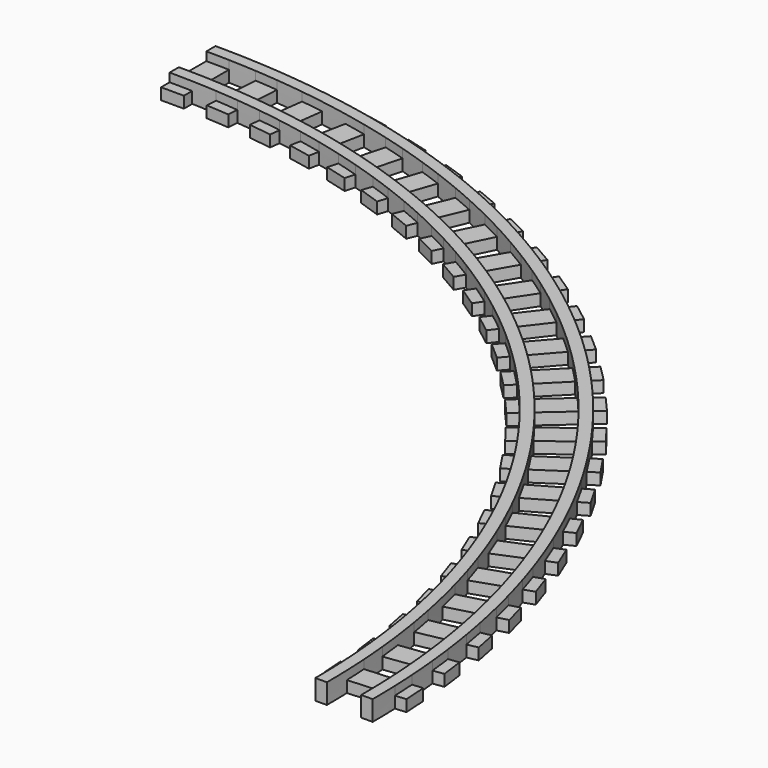
from build123d import *

# Parameters (mm, degrees)
F1_DEPTH = 0.8
F2_DEPTH = 1.4


with BuildPart() as f1:
    # F0 (on Top) → F1 (new body)
    with BuildSketch(Plane.XY):
        with BuildLine():
            ThreePointArc((16.6311172151, 48.993691435), (17.386763269, 48.7306507578), (18.1382513267, 48.4559562805))
            Line((18.1382513267, 48.4559562805), (18.9100588055, 50.729627795))
            ThreePointArc((18.9100588055, 50.729627795), (18.1582983344, 51.0035455811), (17.4025719318, 51.2663237458))
            Line((17.4025719318, 51.2663237458), (16.6311172151, 48.993691435))
        make_face()
        with BuildLine():
            ThreePointArc((9.9358681623, 49.9509824011), (10.7193670612, 49.788726523), (11.5002202458, 49.6141819773))
            Line((11.5002202458, 49.6141819773), (11.6583046084, 50.4089257365))
            ThreePointArc((11.6583046084, 50.4089257365), (10.8773908111, 50.5831812898), (10.093875716, 50.7453400154))
            Line((10.093875716, 50.7453400154), (9.9358681623, 49.9509824011))
        make_face()
        with BuildLine():
            ThreePointArc((50.7453400154, 10.093875716), (50.8953631337, 9.3079466984), (51.0332147669, 8.5197917112))
            Line((51.0332147669, 8.5197917112), (53.3881757978, 8.9882225849))
            ThreePointArc((53.3881757978, 8.9882225849), (53.2495153236, 9.7762251435), (53.0992246884, 10.5620924888))
            Line((53.0992246884, 10.5620924888), (50.7453400154, 10.093875716))
        make_face()
        with BuildLine():
            ThreePointArc((10.093875716, 50.7453400154), (10.8773908111, 50.5831812898), (11.6583046084, 50.4089257365))
            Line((11.6583046084, 50.4089257365), (12.1267354822, 52.7638867673))
            ThreePointArc((12.1267354822, 52.7638867673), (11.3456529805, 52.9373367171), (10.5620924888, 53.0992246884))
            Line((10.5620924888, 53.0992246884), (10.093875716, 50.7453400154))
        make_face()
        with BuildLine():
            ThreePointArc((48.993691435, 16.6311172151), (49.2450154067, 15.8714938755), (49.4845625695, 15.1080749123))
            Line((49.4845625695, 15.1080749123), (51.758234084, 15.8798823911))
            ThreePointArc((51.758234084, 15.8798823911), (51.5179048959, 16.6430446549), (51.2663237458, 17.4025719318))
            Line((51.2663237458, 17.4025719318), (48.993691435, 16.6311172151))
        make_face()
        with BuildLine():
            ThreePointArc((44.8077213791, 25.86975), (45.2024113931, 25.1737534845), (45.5862913757, 24.4717367357))
            Line((45.5862913757, 24.4717367357), (47.66570276, 25.6722854582))
            ThreePointArc((47.66570276, 25.6722854582), (47.2811058581, 26.3738978743), (46.8861823482, 27.06975))
            Line((46.8861823482, 27.06975), (44.8077213791, 25.86975))
        make_face()
        with BuildLine():
            ThreePointArc((34.1142228004, 38.8998157191), (34.7116874142, 38.3676245956), (35.3008508242, 37.8262579611))
            Line((35.3008508242, 37.8262579611), (36.8840043762, 39.6314986018))
            ThreePointArc((36.8840043762, 39.6314986018), (36.2942920622, 40.1722519154), (35.6966527566, 40.704231257))
            Line((35.6966527566, 40.704231257), (34.1142228004, 38.8998157191))
        make_face()
        with BuildLine():
            ThreePointArc((51.2968614051, 6.7533599224), (51.3951610952, 5.9593016578), (51.481169775, 5.1638182427))
            Line((51.481169775, 5.1638182427), (53.8617254985, 5.4772243493))
            ThreePointArc((53.8617254985, 5.4772243493), (53.7748997402, 6.2726085629), (53.6763290723, 7.0666227837))
            Line((53.6763290723, 7.0666227837), (51.2968614051, 6.7533599224))
        make_face()
        with BuildLine():
            ThreePointArc((22.8837956876, 46.4037472105), (23.5986433868, 46.0443252807), (24.3078475358, 45.6738919781))
            Line((24.3078475358, 45.6738919781), (25.3698257798, 47.8273708262))
            ThreePointArc((25.3698257798, 47.8273708262), (24.6602501694, 48.1970696395), (23.9452885441, 48.5562417902))
            Line((23.9452885441, 48.5562417902), (22.8837956876, 46.4037472105))
        make_face()
        with BuildLine():
            ThreePointArc((13.3911679841, 49.9765192893), (14.1623998252, 49.7634634189), (14.9302447677, 49.5385067541))
            Line((14.9302447677, 49.5385067541), (15.5516945156, 51.8577887876))
            ThreePointArc((15.5516945156, 51.8577887876), (14.783628541, 52.0819526075), (14.0123336923, 52.2947412724))
            Line((14.0123336923, 52.2947412724), (13.3911679841, 49.9765192893))
        make_face()
        with BuildLine():
            ThreePointArc((3.3839252048, 51.6287217589), (4.1819031807, 51.5702195655), (4.9788810661, 51.4993844971))
            Line((4.9788810661, 51.4993844971), (5.1359203526, 53.8953410081))
            ThreePointArc((5.1359203526, 53.8953410081), (4.3388803585, 53.9653553447), (3.540892715, 54.0235831747))
            Line((3.540892715, 54.0235831747), (3.3839252048, 51.6287217589))
        make_face()
        with BuildLine():
            ThreePointArc((46.4037472105, 22.8837956876), (46.7520718129, 22.1634753921), (47.0892157868, 21.4378547629))
            Line((47.0892157868, 21.4378547629), (49.2426946349, 22.4998330069))
            ThreePointArc((49.2426946349, 22.4998330069), (48.9048088321, 23.2250970579), (48.5562417902, 23.9452885441))
            Line((48.5562417902, 23.9452885441), (46.4037472105, 22.8837956876))
        make_face()
        with BuildLine():
            ThreePointArc((31.4970119562, 41.04770515), (32.1280043173, 40.5557295439), (32.7513133551, 40.0540551476))
            Line((32.7513133551, 40.0540551476), (34.2130088669, 41.9589738259))
            ThreePointArc((34.2130088669, 41.9589738259), (33.5891922134, 42.4600003144), (32.9580393858, 42.9517531667))
            Line((32.9580393858, 42.9517531667), (31.4970119562, 41.04770515))
        make_face()
        with BuildLine():
            ThreePointArc((38.8998157191, 34.1142228004), (39.4227040594, 33.5085998647), (39.9361645694, 32.8949634403))
            Line((39.9361645694, 32.8949634403), (41.7414052101, 34.4781169923))
            ThreePointArc((41.7414052101, 34.4781169923), (41.2273204377, 35.0912169891), (40.704231257, 35.6966527566))
            Line((40.704231257, 35.6966527566), (38.8998157191, 34.1142228004))
        make_face()
        with BuildLine():
            ThreePointArc((25.86975, 44.8077213791), (26.5595598365, 44.4023157228), (27.2430180278, 43.9862913757))
            Line((27.2430180278, 43.9862913757), (28.4435667503, 46.06570276))
            ThreePointArc((28.4435667503, 46.06570276), (27.759689855, 46.481018485), (27.06975, 46.8861823482))
            Line((27.06975, 46.8861823482), (25.86975, 44.8077213791))
        make_face()
        with BuildLine():
            ThreePointArc((43.0198220057, 28.7449260713), (43.4591873081, 28.0762336998), (43.8881594664, 27.4008269748))
            Line((43.8881594664, 27.4008269748), (45.884599028, 28.7348052418))
            ThreePointArc((45.884599028, 28.7348052418), (45.4549379301, 29.4097616111), (45.0153490753, 30.0782946306))
            Line((45.0153490753, 30.0782946306), (43.0198220057, 28.7449260713))
        make_face()
        with BuildLine():
            ThreePointArc((6.7533599224, 51.2968614051), (7.5458031397, 51.1862942127), (8.3364417991, 51.0634859599))
            Line((8.3364417991, 51.0634859599), (8.6498479057, 53.4440416834))
            ThreePointArc((8.6498479057, 53.4440416834), (7.8590935922, 53.5660350237), (7.0666227837, 53.6763290723))
            Line((7.0666227837, 53.6763290723), (6.7533599224, 51.2968614051))
        make_face()
        with BuildLine():
            ThreePointArc((47.8010650724, 19.7998494489), (48.1015326836, 19.0582898954), (48.3904969466, 18.3121726048))
            Line((48.3904969466, 18.3121726048), (50.6088217316, 19.2310328165))
            ThreePointArc((50.6088217316, 19.2310328165), (50.3190939066, 19.9768428103), (50.0183759504, 20.7182896865))
            Line((50.0183759504, 20.7182896865), (47.8010650724, 19.7998494489))
        make_face()
        with BuildLine():
            ThreePointArc((49.9765192893, 13.3911679841), (50.1776234136, 12.6167336823), (50.3667276984, 11.8392821235))
            Line((50.3667276984, 11.8392821235), (52.686009732, 12.4607318714))
            ThreePointArc((52.686009732, 12.4607318714), (52.4961083073, 13.2379784272), (52.2947412724, 14.0123336923))
            Line((52.2947412724, 14.0123336923), (49.9765192893, 13.3911679841))
        make_face()
        with BuildLine():
            ThreePointArc((51.6287217589, 3.3839252048), (51.6748770866, 2.5851379726), (51.7086745106, 1.7857325117))
            Line((51.7086745106, 1.7857325117), (54.1046310217, 1.9427717982))
            ThreePointArc((54.1046310217, 1.9427717982), (54.0700117805, 2.7421317094), (54.0235831747, 3.540892715))
            Line((54.0235831747, 3.540892715), (51.6287217589, 3.3839252048))
        make_face()
        with BuildLine():
            ThreePointArc((19.7998494489, 47.8010650724), (20.5366739232, 47.4891659689), (21.2685871088, 47.1659099631))
            Line((21.2685871088, 47.1659099631), (22.1874473205, 49.384234748))
            ThreePointArc((22.1874473205, 49.384234748), (21.4552115067, 49.7067335424), (20.7182896865, 50.0183759504))
            Line((20.7182896865, 50.0183759504), (19.7998494489, 47.8010650724))
        make_face()
        with BuildLine():
            ThreePointArc((36.5853513052, 36.5853513052), (37.1467297366, 36.0152235884), (37.6992246306, 35.4364829308))
            Line((37.6992246306, 35.4364829308), (39.3970569162, 37.1343152164))
            ThreePointArc((39.3970569162, 37.1343152164), (38.8439741804, 37.7124797663), (38.28240758, 38.28240758))
            Line((38.28240758, 38.28240758), (36.5853513052, 36.5853513052))
        make_face()
        with BuildLine():
            ThreePointArc((28.7449260713, 43.0198220057), (29.4067441734, 42.5701686321), (30.0615297342, 42.1103347207))
            Line((30.0615297342, 42.1103347207), (31.3955080012, 44.1067742824))
            ThreePointArc((31.3955080012, 44.1067742824), (30.7402582868, 44.5659284735), (30.0782946306, 45.0153490753))
            Line((30.0782946306, 45.0153490753), (28.7449260713, 43.0198220057))
        make_face()
        with BuildLine():
            ThreePointArc((41.04770515, 31.4970119562), (41.5298643112, 30.858487172), (42.0020917204, 30.2125826662))
            Line((42.0020917204, 30.2125826662), (43.9070103987, 31.674278178))
            ThreePointArc((43.9070103987, 31.674278178), (43.4341249795, 32.3196882335), (42.9517531667, 32.9580393858))
            Line((42.9517531667, 32.9580393858), (41.04770515, 31.4970119562))
        make_face()
        with BuildLine():
            ThreePointArc((17.877784521, 47.6886458142), (18.6865502118, 47.377578665), (19.4899064833, 47.0527965614))
            Line((19.4899064833, 47.0527965614), (19.7998494489, 47.8010650724))
            ThreePointArc((19.7998494489, 47.8010650724), (18.9718763763, 48.1356808097), (18.1382513267, 48.4559562805))
            Line((18.1382513267, 48.4559562805), (17.877784521, 47.6886458142))
        make_face()
        with BuildLine():
            ThreePointArc((31.0039638996, 40.4051524126), (31.6348987652, 39.9130968367), (32.2580256231, 39.4111900591))
            Line((32.2580256231, 39.4111900591), (32.7513133551, 40.0540551476))
            ThreePointArc((32.7513133551, 40.0540551476), (32.1280043173, 40.5557295439), (31.4970119562, 41.04770515))
            Line((31.4970119562, 41.04770515), (31.0039638996, 40.4051524126))
        make_face()
        with BuildLine():
            ThreePointArc((53.3881757978, 8.9882225849), (53.5408739863, 8.028715528), (53.6763290723, 7.0666227837))
            Line((53.6763290723, 7.0666227837), (54.4694849614, 7.1710437375))
            ThreePointArc((54.4694849614, 7.1710437375), (54.3302732272, 8.1590484313), (54.1731418966, 9.1443620499))
            Line((54.1731418966, 9.1443620499), (53.3881757978, 8.9882225849))
        make_face()
        with BuildLine():
            ThreePointArc((53.8617254985, 5.4772243493), (53.9513419845, 4.5097847313), (54.0235831747, 3.540892715))
            Line((54.0235831747, 3.540892715), (54.8218703133, 3.5932152183))
            ThreePointArc((54.8218703133, 3.5932152183), (54.7475752407, 4.5882094014), (54.6552229343, 5.5816902686))
            Line((54.6552229343, 5.5816902686), (53.8617254985, 5.4772243493))
        make_face()
        with BuildLine():
            ThreePointArc((13.1815452631, 49.1941966441), (13.9527545885, 48.9810448885), (14.720520147, 48.7558038143))
            Line((14.720520147, 48.7558038143), (14.9302447677, 49.5385067541))
            ThreePointArc((14.9302447677, 49.5385067541), (14.1623998252, 49.7634634189), (13.3911679841, 49.9765192893))
            Line((13.3911679841, 49.9765192893), (13.1815452631, 49.1941966441))
        make_face()
        with BuildLine():
            ThreePointArc((43.2144082401, 26.9506407982), (43.6666795201, 26.2115092786), (44.1063100841, 25.46479))
            Line((44.1063100841, 25.46479), (44.8077213791, 25.86975))
            ThreePointArc((44.8077213791, 25.86975), (44.3545473307, 26.6392565838), (43.8881594664, 27.4008269748))
            Line((43.8881594664, 27.4008269748), (43.2144082401, 26.9506407982))
        make_face()
        with BuildLine():
            ThreePointArc((41.7414052101, 34.4781169923), (42.353399249, 33.7235086002), (42.9517531667, 32.9580393858))
            Line((42.9517531667, 32.9580393858), (43.5864358389, 33.445048529))
            ThreePointArc((43.5864358389, 33.445048529), (42.9718725937, 34.2310798259), (42.3431360603, 35.0058207849))
            Line((42.3431360603, 35.0058207849), (41.7414052101, 34.4781169923))
        make_face()
        with BuildLine():
            ThreePointArc((52.686009732, 12.4607318714), (52.901135746, 11.5132661322), (53.0992246884, 10.5620924888))
            Line((53.0992246884, 10.5620924888), (53.8838529127, 10.7181647464))
            ThreePointArc((53.8838529127, 10.7181647464), (53.6803206428, 11.6949491633), (53.4590831485, 12.6678762691))
            Line((53.4590831485, 12.6678762691), (52.686009732, 12.4607318714))
        make_face()
        with BuildLine():
            ThreePointArc((15.5516945156, 51.8577887876), (16.479786922, 51.5703605112), (17.4025719318, 51.2663237458))
            Line((17.4025719318, 51.2663237458), (17.659723504, 52.0238678494))
            ThreePointArc((17.659723504, 52.0238678494), (16.71203725, 52.3359959417), (15.7588389132, 52.6308622042))
            Line((15.7588389132, 52.6308622042), (15.5516945156, 51.8577887876))
        make_face()
        with BuildLine():
            ThreePointArc((53.0992246884, 10.5620924888), (53.2495153236, 9.7762251435), (53.3881757978, 8.9882225849))
            Line((53.3881757978, 8.9882225849), (54.1731418966, 9.1443620499))
            ThreePointArc((54.1731418966, 9.1443620499), (54.0342275372, 9.9323166841), (53.8838529127, 10.7181647464))
            Line((53.8838529127, 10.7181647464), (53.0992246884, 10.5620924888))
        make_face()
        with BuildLine():
            ThreePointArc((17.4025719318, 51.2663237458), (18.1582983344, 51.0035455811), (18.9100588055, 50.729627795))
            Line((18.9100588055, 50.729627795), (19.1673211117, 51.4874981102))
            ThreePointArc((19.1673211117, 51.4874981102), (18.4154752017, 51.7611720631), (17.659723504, 52.0238678494))
            Line((17.659723504, 52.0238678494), (17.4025719318, 51.2663237458))
        make_face()
        with BuildLine():
            ThreePointArc((11.5002202458, 49.6141819773), (12.3426692445, 49.4113411566), (13.1815452631, 49.1941966441))
            Line((13.1815452631, 49.1941966441), (13.3911679841, 49.9765192893))
            ThreePointArc((13.3911679841, 49.9765192893), (12.5266022179, 50.2002001702), (11.6583046084, 50.4089257365))
            Line((11.6583046084, 50.4089257365), (11.5002202458, 49.6141819773))
        make_face()
        with BuildLine():
            ThreePointArc((8.6498479057, 53.4440416834), (9.6075172714, 53.2802127636), (10.5620924888, 53.0992246884))
            Line((10.5620924888, 53.0992246884), (10.7181647464, 53.8838529127))
            ThreePointArc((10.7181647464, 53.8838529127), (9.7378451883, 54.0696128277), (8.754313825, 54.2375391192))
            Line((8.754313825, 54.2375391192), (8.6498479057, 53.4440416834))
        make_face()
        with BuildLine():
            ThreePointArc((22.5255772316, 45.6773520397), (23.2403841414, 45.3178404598), (23.9494549464, 44.9471436996))
            Line((23.9494549464, 44.9471436996), (24.3078475358, 45.6738919781))
            ThreePointArc((24.3078475358, 45.6738919781), (23.5986433868, 46.0443252807), (22.8837956876, 46.4037472105))
            Line((22.8837956876, 46.4037472105), (22.5255772316, 45.6773520397))
        make_face()
        with BuildLine():
            ThreePointArc((1.6, 54.1158522085), (2.5708603366, 54.0784258035), (3.540892715, 54.0235831747))
            Line((3.540892715, 54.0235831747), (3.5932152183, 54.8218703133))
            ThreePointArc((3.5932152183, 54.8218703133), (2.5970358956, 54.8780836474), (1.6, 54.9161967023))
            Line((1.6, 54.9161967023), (1.6, 54.1158522085))
        make_face()
        with BuildLine():
            ThreePointArc((29.6113435575, 41.4365834945), (30.3120411231, 40.9267917375), (31.0039638996, 40.4051524126))
            Line((31.0039638996, 40.4051524126), (31.4970119562, 41.04770515))
            ThreePointArc((31.4970119562, 41.04770515), (30.7838563075, 41.5852143326), (30.0615297342, 42.1103347207))
            Line((30.0615297342, 42.1103347207), (29.6113435575, 41.4365834945))
        make_face()
        with BuildLine():
            ThreePointArc((8.230674636, 50.2601045961), (9.0845863111, 50.112796874), (9.9358681623, 49.9509824011))
            Line((9.9358681623, 49.9509824011), (10.093875716, 50.7453400154))
            ThreePointArc((10.093875716, 50.7453400154), (9.2165316219, 50.9119966718), (8.3364417991, 51.0634859599))
            Line((8.3364417991, 51.0634859599), (8.230674636, 50.2601045961))
        make_face()
        with BuildLine():
            ThreePointArc((47.6418646951, 18.002078973), (47.9412483031, 17.1889159087), (48.2267537845, 16.3707769633))
            Line((48.2267537845, 16.3707769633), (48.993691435, 16.6311172151))
            ThreePointArc((48.993691435, 16.6311172151), (48.6993482861, 17.4742478166), (48.3904969466, 18.3121726048))
            Line((48.3904969466, 18.3121726048), (47.6418646951, 18.002078973))
        make_face()
        with BuildLine():
            ThreePointArc((19.4899064833, 47.0527965614), (20.226696119, 46.740805332), (20.958493477, 46.4172777115))
            Line((20.958493477, 46.4172777115), (21.2685871088, 47.1659099631))
            ThreePointArc((21.2685871088, 47.1659099631), (20.5366739232, 47.4891659689), (19.7998494489, 47.8010650724))
            Line((19.7998494489, 47.8010650724), (19.4899064833, 47.0527965614))
        make_face()
        with BuildLine():
            ThreePointArc((51.758234084, 15.8798823911), (52.0348667209, 14.9485151632), (52.2947412724, 14.0123336923))
            Line((52.2947412724, 14.0123336923), (53.0674819334, 14.2193889284))
            ThreePointArc((53.0674819334, 14.2193889284), (52.8005006843, 15.1807703276), (52.5161043992, 16.1371446973))
            Line((52.5161043992, 16.1371446973), (51.758234084, 15.8798823911))
        make_face()
        with BuildLine():
            ThreePointArc((50.4938703829, 6.6476441488), (50.5920728704, 5.8535699923), (50.6777884112, 5.0580510796))
            Line((50.6777884112, 5.0580510796), (51.481169775, 5.1638182427))
            ThreePointArc((51.481169775, 5.1638182427), (51.3951610952, 5.9593016578), (51.2968614051, 6.7533599224))
            Line((51.2968614051, 6.7533599224), (50.4938703829, 6.6476441488))
        make_face()
        with BuildLine():
            ThreePointArc((36.8840043762, 39.6314986018), (37.5892588812, 38.9632272407), (38.28240758, 38.28240758))
            Line((38.28240758, 38.28240758), (38.848093005, 38.848093005))
            ThreePointArc((38.848093005, 38.848093005), (38.1361897613, 39.5471830948), (37.4117081689, 40.233229452))
            Line((37.4117081689, 40.233229452), (36.8840043762, 39.6314986018))
        make_face()
        with BuildLine():
            ThreePointArc((4.9258840138, 50.690805731), (5.7876017844, 50.5996619016), (6.6476441488, 50.4938703829))
            Line((6.6476441488, 50.4938703829), (6.7533599224, 51.2968614051))
            ThreePointArc((6.7533599224, 51.2968614051), (5.8669944225, 51.4057801876), (4.9788810661, 51.4993844971))
            Line((4.9788810661, 51.4993844971), (4.9258840138, 50.690805731))
        make_face()
        with BuildLine():
            ThreePointArc((46.3624675083, 21.0794621735), (46.714393522, 20.2876207785), (47.0527965614, 19.4899064833))
            Line((47.0527965614, 19.4899064833), (47.8010650724, 19.7998494489))
            ThreePointArc((47.8010650724, 19.7998494489), (47.4522087551, 20.6219238801), (47.0892157868, 21.4378547629))
            Line((47.0892157868, 21.4378547629), (46.3624675083, 21.0794621735))
        make_face()
        with BuildLine():
            ThreePointArc((52.2947412724, 14.0123336923), (52.4961083073, 13.2379784272), (52.686009732, 12.4607318714))
            Line((52.686009732, 12.4607318714), (53.4590831485, 12.6678762691))
            ThreePointArc((53.4590831485, 12.6678762691), (53.2689315166, 13.4450583981), (53.0674819334, 14.2193889284))
            Line((53.0674819334, 14.2193889284), (52.2947412724, 14.0123336923))
        make_face()
        with BuildLine():
            ThreePointArc((14.0123336923, 52.2947412724), (14.783628541, 52.0819526075), (15.5516945156, 51.8577887876))
            Line((15.5516945156, 51.8577887876), (15.7588389132, 52.6308622042))
            ThreePointArc((15.7588389132, 52.6308622042), (14.9907036302, 52.8547771249), (14.2193889284, 53.0674819334))
            Line((14.2193889284, 53.0674819334), (14.0123336923, 52.2947412724))
        make_face()
        with BuildLine():
            ThreePointArc((33.5802054378, 38.2908856222), (34.177607449, 37.7586184604), (34.7665738706, 37.2170318574))
            Line((34.7665738706, 37.2170318574), (35.3008508242, 37.8262579611))
            ThreePointArc((35.3008508242, 37.8262579611), (34.7116874142, 38.3676245956), (34.1142228004, 38.8998157191))
            Line((34.1142228004, 38.8998157191), (33.5802054378, 38.2908856222))
        make_face()
        with BuildLine():
            ThreePointArc((54.0235831747, 3.540892715), (54.0700117805, 2.7421317094), (54.1046310217, 1.9427717982))
            Line((54.1046310217, 1.9427717982), (54.9032619165, 1.9951168326))
            ThreePointArc((54.9032619165, 1.9951168326), (54.8683847067, 2.794462368), (54.8218703133, 3.5932152183))
            Line((54.8218703133, 3.5932152183), (54.0235831747, 3.540892715))
        make_face()
        with BuildLine():
            ThreePointArc((16.3707769633, 48.2267537845), (17.1263942785, 47.9636189001), (17.877784521, 47.6886458142))
            Line((17.877784521, 47.6886458142), (18.1382513267, 48.4559562805))
            ThreePointArc((18.1382513267, 48.4559562805), (17.386763269, 48.7306507578), (16.6311172151, 48.993691435))
            Line((16.6311172151, 48.993691435), (16.3707769633, 48.2267537845))
        make_face()
        with BuildLine():
            ThreePointArc((28.2949586282, 42.3463981373), (28.9567245882, 41.8966612047), (29.6113435575, 41.4365834945))
            Line((29.6113435575, 41.4365834945), (30.0615297342, 42.1103347207))
            ThreePointArc((30.0615297342, 42.1103347207), (29.4067441734, 42.5701686321), (28.7449260713, 43.0198220057))
            Line((28.7449260713, 43.0198220057), (28.2949586282, 42.3463981373))
        make_face()
        with BuildLine():
            ThreePointArc((40.704231257, 35.6966527566), (41.2273204377, 35.0912169891), (41.7414052101, 34.4781169923))
            Line((41.7414052101, 34.4781169923), (42.3431360603, 35.0058207849))
            ThreePointArc((42.3431360603, 35.0058207849), (41.828855379, 35.6187523354), (41.305703103, 36.2241294087))
            Line((41.305703103, 36.2241294087), (40.704231257, 35.6966527566))
        make_face()
        with BuildLine():
            ThreePointArc((47.0527965614, 19.4899064833), (47.3531743951, 18.7483064217), (47.6418646951, 18.002078973))
            Line((47.6418646951, 18.002078973), (48.3904969466, 18.3121726048))
            ThreePointArc((48.3904969466, 18.3121726048), (48.1015326836, 19.0582898954), (47.8010650724, 19.7998494489))
            Line((47.8010650724, 19.7998494489), (47.0527965614, 19.4899064833))
        make_face()
        with BuildLine():
            ThreePointArc((38.28240758, 38.28240758), (38.8439741804, 37.7124797663), (39.3970569162, 37.1343152164))
            Line((39.3970569162, 37.1343152164), (39.9629859351, 37.7002442353))
            ThreePointArc((39.9629859351, 37.7002442353), (39.4097187268, 38.2782278864), (38.848093005, 38.848093005))
            Line((38.848093005, 38.848093005), (38.28240758, 38.28240758))
        make_face()
        with BuildLine():
            ThreePointArc((42.3463981373, 28.2949586282), (42.7856832901, 27.6262090121), (43.2144082401, 26.9506407982))
            Line((43.2144082401, 26.9506407982), (43.8881594664, 27.4008269748))
            ThreePointArc((43.8881594664, 27.4008269748), (43.4591873081, 28.0762336998), (43.0198220057, 28.7449260713))
            Line((43.0198220057, 28.7449260713), (42.3463981373, 28.2949586282))
        make_face()
        with BuildLine():
            ThreePointArc((42.9517531667, 32.9580393858), (43.4341249795, 32.3196882335), (43.9070103987, 31.674278178))
            Line((43.9070103987, 31.674278178), (44.5419663763, 32.1614970358))
            ThreePointArc((44.5419663763, 32.1614970358), (44.0688744508, 32.8067518186), (43.5864358389, 33.445048529))
            Line((43.5864358389, 33.445048529), (42.9517531667, 32.9580393858))
        make_face()
        with BuildLine():
            ThreePointArc((3.540892715, 54.0235831747), (4.3388803585, 53.9653553447), (5.1359203526, 53.8953410081))
            Line((5.1359203526, 53.8953410081), (5.1882653869, 54.693971903))
            ThreePointArc((5.1882653869, 54.693971903), (4.391205974, 54.7637286015), (3.5932152183, 54.8218703133))
            Line((3.5932152183, 54.8218703133), (3.540892715, 54.0235831747))
        make_face()
        with BuildLine():
            ThreePointArc((37.1262463114, 34.8635046116), (37.7140247317, 34.2268090466), (38.2908856222, 33.5802054378))
            Line((38.2908856222, 33.5802054378), (38.8998157191, 34.1142228004))
            ThreePointArc((38.8998157191, 34.1142228004), (38.3052259957, 34.7805336599), (37.6992246306, 35.4364829308))
            Line((37.6992246306, 35.4364829308), (37.1262463114, 34.8635046116))
        make_face()
        with BuildLine():
            ThreePointArc((51.2663237458, 17.4025719318), (51.5179048959, 16.6430446549), (51.758234084, 15.8798823911))
            Line((51.758234084, 15.8798823911), (52.5161043992, 16.1371446973))
            ThreePointArc((52.5161043992, 16.1371446973), (52.2755297533, 16.9002263079), (52.0238678494, 17.659723504))
            Line((52.0238678494, 17.659723504), (51.2663237458, 17.4025719318))
        make_face()
        with BuildLine():
            ThreePointArc((53.6763290723, 7.0666227837), (53.7748997402, 6.2726085629), (53.8617254985, 5.4772243493))
            Line((53.8617254985, 5.4772243493), (54.6552229343, 5.5816902686))
            ThreePointArc((54.6552229343, 5.5816902686), (54.5681406999, 6.3770432652), (54.4694849614, 7.1710437375))
            Line((54.4694849614, 7.1710437375), (53.6763290723, 7.0666227837))
        make_face()
        with BuildLine():
            ThreePointArc((48.7172521032, 14.8476081066), (48.962811299, 14.0166054621), (49.1941966441, 13.1815452631))
            Line((49.1941966441, 13.1815452631), (49.9765192893, 13.3911679841))
            ThreePointArc((49.9765192893, 13.3911679841), (49.7379497314, 14.2517443413), (49.4845625695, 15.1080749123))
            Line((49.4845625695, 15.1080749123), (48.7172521032, 14.8476081066))
        make_face()
        with BuildLine():
            ThreePointArc((31.3955080012, 44.1067742824), (32.1819558723, 43.5362742605), (32.9580393858, 42.9517531667))
            Line((32.9580393858, 42.9517531667), (33.445048529, 43.5864358389))
            ThreePointArc((33.445048529, 43.5864358389), (32.6479861489, 44.1866230965), (31.8401555782, 44.7722364084))
            Line((31.8401555782, 44.7722364084), (31.3955080012, 44.1067742824))
        make_face()
        with BuildLine():
            ThreePointArc((45.884599028, 28.7348052418), (46.392861213, 27.9067713776), (46.8861823482, 27.06975))
            Line((46.8861823482, 27.06975), (47.5790026712, 27.46975))
            ThreePointArc((47.5790026712, 27.46975), (47.0722947718, 28.3292732904), (46.5500611541, 29.1794528188))
            Line((46.5500611541, 29.1794528188), (45.884599028, 28.7348052418))
        make_face()
        with BuildLine():
            ThreePointArc((3.3309539024, 50.8205358598), (4.1289285014, 50.7619352311), (4.9258840138, 50.690805731))
            Line((4.9258840138, 50.690805731), (4.9788810661, 51.4993844971))
            ThreePointArc((4.9788810661, 51.4993844971), (4.1819031807, 51.5702195655), (3.3839252048, 51.6287217589))
            Line((3.3839252048, 51.6287217589), (3.3309539024, 50.8205358598))
        make_face()
        with BuildLine():
            ThreePointArc((25.46479, 44.1063100841), (26.154553271, 43.7008176373), (26.8378611728, 43.2845391178))
            Line((26.8378611728, 43.2845391178), (27.2430180278, 43.9862913757))
            ThreePointArc((27.2430180278, 43.9862913757), (26.5595598365, 44.4023157228), (25.86975, 44.8077213791))
            Line((25.86975, 44.8077213791), (25.46479, 44.1063100841))
        make_face()
        with BuildLine():
            ThreePointArc((27.06975, 46.8861823482), (27.759689855, 46.481018485), (28.4435667503, 46.06570276))
            Line((28.4435667503, 46.06570276), (28.8437389972, 46.7588214234))
            ThreePointArc((28.8437389972, 46.7588214234), (28.1597307352, 47.1739146687), (27.46975, 47.5790026712))
            Line((27.46975, 47.5790026712), (27.06975, 46.8861823482))
        make_face()
        with BuildLine():
            ThreePointArc((49.5840247586, 11.6295575029), (49.7747080199, 10.784273759), (49.9509824011, 9.9358681623))
            Line((49.9509824011, 9.9358681623), (50.7453400154, 10.093875716))
            ThreePointArc((50.7453400154, 10.093875716), (50.5635656399, 10.9682127088), (50.3667276984, 11.8392821235))
            Line((50.3667276984, 11.8392821235), (49.5840247586, 11.6295575029))
        make_face()
        with BuildLine():
            ThreePointArc((28.4435667503, 46.06570276), (29.2656432628, 45.5478603742), (30.0782946306, 45.0153490753))
            Line((30.0782946306, 45.0153490753), (30.522750817, 45.6805247651))
            ThreePointArc((30.522750817, 45.6805247651), (29.6881408838, 46.2272966018), (28.8437389972, 46.7588214234))
            Line((28.8437389972, 46.7588214234), (28.4435667503, 46.06570276))
        make_face()
        with BuildLine():
            ThreePointArc((33.445048529, 43.5864358389), (34.0762517889, 43.0947528624), (34.7002277247, 42.5939298035))
            Line((34.7002277247, 42.5939298035), (35.1649460319, 43.1995624926))
            Line((35.1649460319, 43.1995624926), (33.8955806874, 44.173580779))
            Line((33.8955806874, 44.173580779), (33.445048529, 43.5864358389))
        make_face()
        with BuildLine():
            ThreePointArc((25.3698257798, 47.8273708262), (26.2240106759, 47.3644035571), (27.06975, 46.8861823482))
            Line((27.06975, 46.8861823482), (27.46975, 47.5790026712))
            ThreePointArc((27.46975, 47.5790026712), (26.6011664416, 48.0700177262), (25.7238090977, 48.5451779866))
            Line((25.7238090977, 48.5451779866), (25.3698257798, 47.8273708262))
        make_face()
        with BuildLine():
            ThreePointArc((45.0153490753, 30.0782946306), (45.4549379301, 29.4097616111), (45.884599028, 28.7348052418))
            Line((45.884599028, 28.7348052418), (46.5500611541, 29.1794528188))
            ThreePointArc((46.5500611541, 29.1794528188), (46.1201838366, 29.8542677539), (45.6805247651, 30.522750817))
            Line((45.6805247651, 30.522750817), (45.0153490753, 30.0782946306))
        make_face()
        with BuildLine():
            ThreePointArc((48.2267537845, 16.3707769633), (48.4779855216, 15.611119074), (48.7172521032, 14.8476081066))
            Line((48.7172521032, 14.8476081066), (49.4845625695, 15.1080749123))
            ThreePointArc((49.4845625695, 15.1080749123), (49.2450154067, 15.8714938755), (48.993691435, 16.6311172151))
            Line((48.993691435, 16.6311172151), (48.2267537845, 16.3707769633))
        make_face()
        with BuildLine():
            Line((48.0308593319, 14.6146091571), (48.7172521032, 14.8476081066))
            ThreePointArc((48.7172521032, 14.8476081066), (48.4779855216, 15.611119074), (48.2267537845, 16.3707769633))
            Line((48.2267537845, 16.3707769633), (47.5165561874, 16.1296973643))
            Line((47.5165561874, 16.1296973643), (48.0308593319, 14.6146091571))
        make_face()
        with BuildLine():
            ThreePointArc((44.8845391178, 24.0665798807), (45.287500536, 23.2994509415), (45.6773520397, 22.5255772316))
            Line((45.6773520397, 22.5255772316), (46.4037472105, 22.8837956876))
            ThreePointArc((46.4037472105, 22.8837956876), (46.0018715811, 23.6812936995), (45.5862913757, 24.4717367357))
            Line((45.5862913757, 24.4717367357), (44.8845391178, 24.0665798807))
        make_face()
        with BuildLine():
            ThreePointArc((39.3970569162, 37.1343152164), (40.057094379, 36.421348824), (40.704231257, 35.6966527566))
            Line((40.704231257, 35.6966527566), (41.305703103, 36.2241294087))
            ThreePointArc((41.305703103, 36.2241294087), (40.6410467783, 36.9682833928), (39.9629859351, 37.7002442353))
            Line((39.9629859351, 37.7002442353), (39.3970569162, 37.1343152164))
        make_face()
        with BuildLine():
            ThreePointArc((1.6, 50.9044410536), (2.4658338584, 50.8698514089), (3.3309539024, 50.8205358598))
            Line((3.3309539024, 50.8205358598), (3.3839252048, 51.6287217589))
            ThreePointArc((3.3839252048, 51.6287217589), (2.4923338523, 51.6794362607), (1.6, 51.7147547635))
            Line((1.6, 51.7147547635), (1.6, 50.9044410536))
        make_face()
        with BuildLine():
            ThreePointArc((22.1874473205, 49.384234748), (23.0700828493, 48.9781250925), (23.9452885441, 48.5562417902))
            Line((23.9452885441, 48.5562417902), (24.2991194963, 49.2737399834))
            ThreePointArc((24.2991194963, 49.2737399834), (23.4002817209, 49.7068956547), (22.4937258985, 50.1236566449))
            Line((22.4937258985, 50.1236566449), (22.1874473205, 49.384234748))
        make_face()
        with BuildLine():
            ThreePointArc((50.6777884112, 5.0580510796), (50.7565086823, 4.1951096953), (50.8205358598, 3.3309539024))
            Line((50.8205358598, 3.3309539024), (51.6287217589, 3.3839252048))
            ThreePointArc((51.6287217589, 3.3839252048), (51.5626263668, 4.2745084405), (51.481169775, 5.1638182427))
            Line((51.481169775, 5.1638182427), (50.6777884112, 5.0580510796))
        make_face()
        with BuildLine():
            ThreePointArc((50.0183759504, 20.7182896865), (50.3190939066, 19.9768428103), (50.6088217316, 19.2310328165))
            Line((50.6088217316, 19.2310328165), (51.3482436284, 19.5373113945))
            ThreePointArc((51.3482436284, 19.5373113945), (51.0582761461, 20.2830248542), (50.7574795764, 21.0244364324))
            Line((50.7574795764, 21.0244364324), (50.0183759504, 20.7182896865))
        make_face()
        with BuildLine():
            ThreePointArc((0, 50.92958), (0.8000987387, 50.9232948756), (1.6, 50.9044410536))
            Line((1.6, 50.9044410536), (1.6, 51.7147547635))
            ThreePointArc((1.6, 51.7147547635), (0.8000956703, 51.733313321), (0, 51.7395))
            Line((0, 51.7395), (0, 50.92958))
        make_face()
        with BuildLine():
            ThreePointArc((50.2384710077, 8.3617073485), (50.3734617996, 7.50576214), (50.4938703829, 6.6476441488))
            Line((50.4938703829, 6.6476441488), (51.2968614051, 6.7533599224))
            ThreePointArc((51.2968614051, 6.7533599224), (51.1726605978, 7.6377135055), (51.0332147669, 8.5197917112))
            Line((51.0332147669, 8.5197917112), (50.2384710077, 8.3617073485))
        make_face()
        with BuildLine():
            ThreePointArc((6.6476441488, 50.4938703829), (7.4400775585, 50.3832051869), (8.230674636, 50.2601045961))
            Line((8.230674636, 50.2601045961), (8.3364417991, 51.0634859599))
            ThreePointArc((8.3364417991, 51.0634859599), (7.5458031397, 51.1862942127), (6.7533599224, 51.2968614051))
            Line((6.7533599224, 51.2968614051), (6.6476441488, 50.4938703829))
        make_face()
        with BuildLine():
            ThreePointArc((54.1046310217, 1.9427717982), (54.1307820535, 0.9715423441), (54.1395, 0))
            Line((54.1395, 0), (54.9395, 0))
            ThreePointArc((54.9395, 0), (54.9304397321, 0.9977229543), (54.9032619165, 1.9951168326))
            Line((54.9032619165, 1.9951168326), (54.1046310217, 1.9427717982))
        make_face()
        with BuildLine():
            ThreePointArc((41.3592266319, 29.7192949342), (41.8588710787, 29.011325909), (42.3463981373, 28.2949586282))
            Line((42.3463981373, 28.2949586282), (43.0198220057, 28.7449260713))
            ThreePointArc((43.0198220057, 28.7449260713), (42.5172900992, 29.4831460816), (42.0020917204, 30.2125826662))
            Line((42.0020917204, 30.2125826662), (41.3592266319, 29.7192949342))
        make_face()
        with BuildLine():
            ThreePointArc((50.7574795764, 21.0244364324), (51.0582761461, 20.2830248542), (51.3482436284, 19.5373113945))
            Line((51.3482436284, 19.5373113945), (52.0535178326, 19.829445535))
            Line((52.0535178326, 19.829445535), (51.4412243408, 21.307652787))
            Line((51.4412243408, 21.307652787), (50.7574795764, 21.0244364324))
        make_face()
        with BuildLine():
            ThreePointArc((7.1710437375, 54.4694849614), (7.9635232838, 54.3592766431), (8.754313825, 54.2375391192))
            Line((8.754313825, 54.2375391192), (8.85395534, 54.9943915669))
            Line((8.85395534, 54.9943915669), (7.2676435618, 55.2032334745))
            Line((7.2676435618, 55.2032334745), (7.1710437375, 54.4694849614))
        make_face()
        with BuildLine():
            ThreePointArc((0, 54.1395), (0.800087373, 54.1335877293), (1.6, 54.1158522085))
            Line((1.6, 54.1158522085), (1.6, 54.9161967023))
            ThreePointArc((1.6, 54.9161967023), (0.8000848461, 54.9336738667), (0, 54.9395))
            Line((0, 54.9395), (0, 54.1395))
        make_face()
        with BuildLine():
            ThreePointArc((32.2580256231, 39.4111900591), (32.9238809653, 38.856661992), (33.5802054378, 38.2908856222))
            Line((33.5802054378, 38.2908856222), (34.1142228004, 38.8998157191))
            ThreePointArc((34.1142228004, 38.8998157191), (33.4377488552, 39.4828166643), (32.7513133551, 40.0540551476))
            Line((32.7513133551, 40.0540551476), (32.2580256231, 39.4111900591))
        make_face()
        with BuildLine():
            ThreePointArc((38.848093005, 38.848093005), (39.4097187268, 38.2782278864), (39.9629859351, 37.7002442353))
            Line((39.9629859351, 37.7002442353), (40.5027794415, 38.2400377417))
            Line((40.5027794415, 38.2400377417), (39.3714085916, 39.3714085916))
            Line((39.3714085916, 39.3714085916), (38.848093005, 38.848093005))
        make_face()
        with BuildLine():
            ThreePointArc((40.4051524126, 31.0039638996), (40.8872353397, 30.3653767514), (41.3592266319, 29.7192949342))
            Line((41.3592266319, 29.7192949342), (42.0020917204, 30.2125826662))
            ThreePointArc((42.0020917204, 30.2125826662), (41.5298643112, 30.858487172), (41.04770515, 31.4970119562))
            Line((41.04770515, 31.4970119562), (40.4051524126, 31.0039638996))
        make_face()
        with BuildLine():
            ThreePointArc((50.6088217316, 19.2310328165), (50.945776408, 18.3197523574), (51.2663237458, 17.4025719318))
            Line((51.2663237458, 17.4025719318), (52.0238678494, 17.659723504))
            ThreePointArc((52.0238678494, 17.659723504), (51.6945808757, 18.6015851027), (51.3482436284, 19.5373113945))
            Line((51.3482436284, 19.5373113945), (50.6088217316, 19.2310328165))
        make_face()
        with BuildLine():
            ThreePointArc((46.8861823482, 27.06975), (47.2811058581, 26.3738978743), (47.66570276, 25.6722854582))
            Line((47.66570276, 25.6722854582), (48.3588214234, 26.0724577051))
            ThreePointArc((48.3588214234, 26.0724577051), (47.9739995148, 26.7739431314), (47.5790026712, 27.46975))
            Line((47.5790026712, 27.46975), (46.8861823482, 27.06975))
        make_face()
        with BuildLine():
            ThreePointArc((54.4694849614, 7.1710437375), (54.5681406999, 6.3770432652), (54.6552229343, 5.5816902686))
            Line((54.6552229343, 5.5816902686), (55.412075382, 5.6813317836))
            Line((55.412075382, 5.6813317836), (55.2032334745, 7.2676435618))
            Line((55.2032334745, 7.2676435618), (54.4694849614, 7.1710437375))
        make_face()
        with BuildLine():
            ThreePointArc((38.2908856222, 33.5802054378), (38.8137019705, 32.9745152857), (39.3269384657, 32.3606864867))
            Line((39.3269384657, 32.3606864867), (39.9361645694, 32.8949634403))
            ThreePointArc((39.9361645694, 32.8949634403), (39.4227040594, 33.5085998647), (38.8998157191, 34.1142228004))
            Line((38.8998157191, 34.1142228004), (38.2908856222, 33.5802054378))
        make_face()
        with BuildLine():
            ThreePointArc((48.5562417902, 23.9452885441), (48.9048088321, 23.2250970579), (49.2426946349, 22.4998330069))
            Line((49.2426946349, 22.4998330069), (49.9605017953, 22.8538163248))
            ThreePointArc((49.9605017953, 22.8538163248), (49.6223831619, 23.578968374), (49.2737399834, 24.2991194963))
            Line((49.2737399834, 24.2991194963), (48.5562417902, 23.9452885441))
        make_face()
        with BuildLine():
            ThreePointArc((14.2193889284, 53.0674819334), (14.9907036302, 52.8547771249), (15.7588389132, 52.6308622042))
            Line((15.7588389132, 52.6308622042), (15.9564170494, 53.3682338468))
            Line((15.9564170494, 53.3682338468), (14.4109357273, 53.7823443189))
            Line((14.4109357273, 53.7823443189), (14.2193889284, 53.0674819334))
        make_face()
        with BuildLine():
            ThreePointArc((34.7665738706, 37.2170318574), (35.3947356946, 36.6201420545), (36.012651381, 36.012651381))
            Line((36.012651381, 36.012651381), (36.5853513052, 36.5853513052))
            ThreePointArc((36.5853513052, 36.5853513052), (35.9484558289, 37.2113475135), (35.3008508242, 37.8262579611))
            Line((35.3008508242, 37.8262579611), (34.7665738706, 37.2170318574))
        make_face()
        with BuildLine():
            ThreePointArc((35.6966527566, 40.704231257), (36.2942920622, 40.1722519154), (36.8840043762, 39.6314986018))
            Line((36.8840043762, 39.6314986018), (37.4117081689, 40.233229452))
            ThreePointArc((37.4117081689, 40.233229452), (36.8218236087, 40.773790189), (36.2241294087, 41.305703103))
            Line((36.2241294087, 41.305703103), (35.6966527566, 40.704231257))
        make_face()
        with BuildLine():
            ThreePointArc((49.9509824011, 9.9358681623), (50.1009095642, 9.1499169296), (50.2384710077, 8.3617073485))
            Line((50.2384710077, 8.3617073485), (51.0332147669, 8.5197917112))
            ThreePointArc((51.0332147669, 8.5197917112), (50.8953631337, 9.3079466984), (50.7453400154, 10.093875716))
            Line((50.7453400154, 10.093875716), (49.9509824011, 9.9358681623))
        make_face()
        with BuildLine():
            ThreePointArc((30.0782946306, 45.0153490753), (30.7402582868, 44.5659284735), (31.3955080012, 44.1067742824))
            Line((31.3955080012, 44.1067742824), (31.8401555782, 44.7722364084))
            ThreePointArc((31.8401555782, 44.7722364084), (31.1847602275, 45.2311771879), (30.522750817, 45.6805247651))
            Line((30.522750817, 45.6805247651), (30.0782946306, 45.0153490753))
        make_face()
        with BuildLine():
            ThreePointArc((43.5864358389, 33.445048529), (44.0688744508, 32.8067518186), (44.5419663763, 32.1614970358))
            Line((44.5419663763, 32.1614970358), (45.1475990654, 32.6262153429))
            Line((45.1475990654, 32.6262153429), (44.173580779, 33.8955806874))
            Line((44.173580779, 33.8955806874), (43.5864358389, 33.445048529))
        make_face()
        with BuildLine():
            ThreePointArc((18.9100588055, 50.729627795), (19.8173653862, 50.382114777), (20.7182896865, 50.0183759504))
            Line((20.7182896865, 50.0183759504), (21.0244364324, 50.7574795764))
            ThreePointArc((21.0244364324, 50.7574795764), (20.0991934014, 51.130921025), (19.1673211117, 51.4874981102))
            Line((19.1673211117, 51.4874981102), (18.9100588055, 50.729627795))
        make_face()
        with BuildLine():
            ThreePointArc((23.9494549464, 44.9471436996), (24.710699124, 44.5331726669), (25.46479, 44.1063100841))
            Line((25.46479, 44.1063100841), (25.86975, 44.8077213791))
            ThreePointArc((25.86975, 44.8077213791), (25.0925364699, 45.2475466048), (24.3078475358, 45.6738919781))
            Line((24.3078475358, 45.6738919781), (23.9494549464, 44.9471436996))
        make_face()
        with BuildLine():
            ThreePointArc((50.9000957445, 1.7327354594), (50.9222084027, 0.8664931468), (50.92958, 0))
            Line((50.92958, 0), (51.7395, 0))
            ThreePointArc((51.7395, 0), (51.7317930537, 0.8929992741), (51.7086745106, 1.7857325117))
            Line((51.7086745106, 1.7857325117), (50.9000957445, 1.7327354594))
        make_face()
        with BuildLine():
            ThreePointArc((27.46975, 47.5790026712), (28.1597307352, 47.1739146687), (28.8437389972, 46.7588214234))
            Line((28.8437389972, 46.7588214234), (29.2254306461, 47.419930752))
            Line((29.2254306461, 47.419930752), (27.83979, 48.219930752))
            Line((27.83979, 48.219930752), (27.46975, 47.5790026712))
        make_face()
        with BuildLine():
            ThreePointArc((23.9452885441, 48.5562417902), (24.6602501694, 48.1970696395), (25.3698257798, 47.8273708262))
            Line((25.3698257798, 47.8273708262), (25.7238090977, 48.5451779866))
            ThreePointArc((25.7238090977, 48.5451779866), (25.0141169528, 48.9146462046), (24.2991194963, 49.2737399834))
            Line((24.2991194963, 49.2737399834), (23.9452885441, 48.5562417902))
        make_face()
        with BuildLine():
            ThreePointArc((45.6805247651, 30.522750817), (46.1201838366, 29.8542677539), (46.5500611541, 29.1794528188))
            Line((46.5500611541, 29.1794528188), (47.1847911686, 29.6035658553))
            Line((47.1847911686, 29.6035658553), (46.2958787958, 30.933917235))
            Line((46.2958787958, 30.933917235), (45.6805247651, 30.522750817))
        make_face()
        with BuildLine():
            ThreePointArc((49.1941966441, 13.1815452631), (49.3952064716, 12.4070825179), (49.5840247586, 11.6295575029))
            Line((49.5840247586, 11.6295575029), (50.3667276984, 11.8392821235))
            ThreePointArc((50.3667276984, 11.8392821235), (50.1776234136, 12.6167336823), (49.9765192893, 13.3911679841))
            Line((49.9765192893, 13.3911679841), (49.1941966441, 13.1815452631))
        make_face()
        with BuildLine():
            ThreePointArc((20.958493477, 46.4172777115), (21.7451827734, 46.053980774), (22.5255772316, 45.6773520397))
            Line((22.5255772316, 45.6773520397), (22.8837956876, 46.4037472105))
            ThreePointArc((22.8837956876, 46.4037472105), (22.0794802852, 46.7917985397), (21.2685871088, 47.1659099631))
            Line((21.2685871088, 47.1659099631), (20.958493477, 46.4172777115))
        make_face()
        with BuildLine():
            ThreePointArc((7.0666227837, 53.6763290723), (7.8590935922, 53.5660350237), (8.6498479057, 53.4440416834))
            Line((8.6498479057, 53.4440416834), (8.754313825, 54.2375391192))
            ThreePointArc((8.754313825, 54.2375391192), (7.9635232838, 54.3592766431), (7.1710437375, 54.4694849614))
            Line((7.1710437375, 54.4694849614), (7.0666227837, 53.6763290723))
        make_face()
        with BuildLine():
            ThreePointArc((36.012651381, 36.012651381), (36.5739623706, 35.4424518831), (37.1262463114, 34.8635046116))
            Line((37.1262463114, 34.8635046116), (37.6992246306, 35.4364829308))
            ThreePointArc((37.6992246306, 35.4364829308), (37.1467297366, 36.0152235884), (36.5853513052, 36.5853513052))
            Line((36.5853513052, 36.5853513052), (36.012651381, 36.012651381))
        make_face()
        with BuildLine():
            ThreePointArc((54.8218703133, 3.5932152183), (54.8683847067, 2.794462368), (54.9032619165, 1.9951168326))
            Line((54.9032619165, 1.9951168326), (55.6650107519, 2.045044489))
            Line((55.6650107519, 2.045044489), (55.5603657452, 3.6416187662))
            Line((55.5603657452, 3.6416187662), (54.8218703133, 3.5932152183))
        make_face()
        with BuildLine():
            ThreePointArc((0, 51.7395), (0.8000956703, 51.733313321), (1.6, 51.7147547635))
            Line((1.6, 51.7147547635), (1.6, 54.1158522085))
            ThreePointArc((1.6, 54.1158522085), (0.800087373, 54.1335877293), (0, 54.1395))
            Line((0, 54.1395), (0, 51.7395))
        make_face()
        with BuildLine():
            ThreePointArc((26.8378611728, 43.2845391178), (27.5704004673, 42.8216666776), (28.2949586282, 42.3463981373))
            Line((28.2949586282, 42.3463981373), (28.7449260713, 43.0198220057))
            ThreePointArc((28.7449260713, 43.0198220057), (27.9981425611, 43.5095377288), (27.2430180278, 43.9862913757))
            Line((27.2430180278, 43.9862913757), (26.8378611728, 43.2845391178))
        make_face()
        with BuildLine():
            ThreePointArc((32.9580393858, 42.9517531667), (33.5891922134, 42.4600003144), (34.2130088669, 41.9589738259))
            Line((34.2130088669, 41.9589738259), (34.7002277247, 42.5939298035))
            ThreePointArc((34.7002277247, 42.5939298035), (34.0762517889, 43.0947528624), (33.445048529, 43.5864358389))
            Line((33.445048529, 43.5864358389), (32.9580393858, 42.9517531667))
        make_face()
        with BuildLine():
            ThreePointArc((43.9070103987, 31.674278178), (44.4683403612, 30.8812591352), (45.0153490753, 30.0782946306))
            Line((45.0153490753, 30.0782946306), (45.6805247651, 30.522750817))
            ThreePointArc((45.6805247651, 30.522750817), (45.1186862534, 31.3472935198), (44.5419663763, 32.1614970358))
            Line((44.5419663763, 32.1614970358), (43.9070103987, 31.674278178))
        make_face()
        with BuildLine():
            ThreePointArc((5.1359203526, 53.8953410081), (6.1022541987, 53.7944974318), (7.0666227837, 53.6763290723))
            Line((7.0666227837, 53.6763290723), (7.1710437375, 54.4694849614))
            ThreePointArc((7.1710437375, 54.4694849614), (6.1806738391, 54.5907311835), (5.1882653869, 54.693971903))
            Line((5.1882653869, 54.693971903), (5.1359203526, 53.8953410081))
        make_face()
        with BuildLine():
            ThreePointArc((49.2426946349, 22.4998330069), (49.6385284591, 21.6125415595), (50.0183759504, 20.7182896865))
            Line((50.0183759504, 20.7182896865), (50.7574795764, 21.0244364324))
            ThreePointArc((50.7574795764, 21.0244364324), (50.3672969356, 21.9427450346), (49.9605017953, 22.8538163248))
            Line((49.9605017953, 22.8538163248), (49.2426946349, 22.4998330069))
        make_face()
        with BuildLine():
            ThreePointArc((53.0674819334, 14.2193889284), (53.2689315166, 13.4450583981), (53.4590831485, 12.6678762691))
            Line((53.4590831485, 12.6678762691), (54.1964547911, 12.8654544052))
            Line((54.1964547911, 12.8654544052), (53.7823443189, 14.4109357273))
            Line((53.7823443189, 14.4109357273), (53.0674819334, 14.2193889284))
        make_face()
        with BuildLine():
            ThreePointArc((41.305703103, 36.2241294087), (41.828855379, 35.6187523354), (42.3431360603, 35.0058207849))
            Line((42.3431360603, 35.0058207849), (42.9170780119, 35.5091543676))
            Line((42.9170780119, 35.5091543676), (41.8621247077, 36.7120980595))
            Line((41.8621247077, 36.7120980595), (41.305703103, 36.2241294087))
        make_face()
        with BuildLine():
            ThreePointArc((12.1267354822, 52.7638867673), (13.0716394802, 52.5377740445), (14.0123336923, 52.2947412724))
            Line((14.0123336923, 52.2947412724), (14.2193889284, 53.0674819334))
            ThreePointArc((14.2193889284, 53.0674819334), (13.2533175895, 53.3169600889), (12.2828749472, 53.5488528662))
            Line((12.2828749472, 53.5488528662), (12.1267354822, 52.7638867673))
        make_face()
        with BuildLine():
            ThreePointArc((34.2130088669, 41.9589738259), (34.9604604061, 41.3382591366), (35.6966527566, 40.704231257))
            Line((35.6966527566, 40.704231257), (36.2241294087, 41.305703103))
            ThreePointArc((36.2241294087, 41.305703103), (35.468027725, 41.9567356874), (34.7002277247, 42.5939298035))
            Line((34.7002277247, 42.5939298035), (34.2130088669, 41.9589738259))
        make_face()
        with BuildLine():
            ThreePointArc((47.66570276, 25.6722854582), (48.1187207108, 24.8127825406), (48.5562417902, 23.9452885441))
            Line((48.5562417902, 23.9452885441), (49.2737399834, 24.2991194963))
            ThreePointArc((49.2737399834, 24.2991194963), (48.8243324974, 25.1899427636), (48.3588214234, 26.0724577051))
            Line((48.3588214234, 26.0724577051), (47.66570276, 25.6722854582))
        make_face()
        with BuildLine():
            ThreePointArc((44.1063100841, 25.46479), (44.500916376, 24.7687416045), (44.8845391178, 24.0665798807))
            Line((44.8845391178, 24.0665798807), (45.5862913757, 24.4717367357))
            ThreePointArc((45.5862913757, 24.4717367357), (45.2024113931, 25.1737534845), (44.8077213791, 25.86975))
            Line((44.8077213791, 25.86975), (44.1063100841, 25.46479))
        make_face()
        with BuildLine():
            ThreePointArc((52.0238678494, 17.659723504), (52.2755297533, 16.9002263079), (52.5161043992, 16.1371446973))
            Line((52.5161043992, 16.1371446973), (53.2389750441, 16.3825262163))
            Line((53.2389750441, 16.3825262163), (52.7246718996, 17.8976144235))
            Line((52.7246718996, 17.8976144235), (52.0238678494, 17.659723504))
        make_face()
        with BuildLine():
            ThreePointArc((50.8205358598, 3.3309539024), (50.8665931535, 2.5321571697), (50.9000957445, 1.7327354594))
            Line((50.9000957445, 1.7327354594), (51.7086745106, 1.7857325117))
            ThreePointArc((51.7086745106, 1.7857325117), (51.6748770866, 2.5851379726), (51.6287217589, 3.3839252048))
            Line((51.6287217589, 3.3839252048), (50.8205358598, 3.3309539024))
        make_face()
        with BuildLine():
            ThreePointArc((10.5620924888, 53.0992246884), (11.3456529805, 52.9373367171), (12.1267354822, 52.7638867673))
            Line((12.1267354822, 52.7638867673), (12.2828749472, 53.5488528662))
            ThreePointArc((12.2828749472, 53.5488528662), (11.5017395643, 53.7220499166), (10.7181647464, 53.8838529127))
            Line((10.7181647464, 53.8838529127), (10.5620924888, 53.0992246884))
        make_face()
        with BuildLine():
            ThreePointArc((20.7182896865, 50.0183759504), (21.4552115067, 49.7067335424), (22.1874473205, 49.384234748))
            Line((22.1874473205, 49.384234748), (22.4937258985, 50.1236566449))
            ThreePointArc((22.4937258985, 50.1236566449), (21.7613888813, 50.445917716), (21.0244364324, 50.7574795764))
            Line((21.0244364324, 50.7574795764), (20.7182896865, 50.0183759504))
        make_face()
        with BuildLine():
            ThreePointArc((17.659723504, 52.0238678494), (18.4154752017, 51.7611720631), (19.1673211117, 51.4874981102))
            Line((19.1673211117, 51.4874981102), (19.4127026307, 52.2103687551))
            Line((19.4127026307, 52.2103687551), (17.8976144235, 52.7246718996))
            Line((17.8976144235, 52.7246718996), (17.659723504, 52.0238678494))
        make_face()
        with BuildLine():
            ThreePointArc((53.8838529127, 10.7181647464), (54.0342275372, 9.9323166841), (54.1731418966, 9.1443620499))
            Line((54.1731418966, 9.1443620499), (54.9218569983, 9.2932907433))
            Line((54.9218569983, 9.2932907433), (54.609712483, 10.8625471919))
            Line((54.609712483, 10.8625471919), (53.8838529127, 10.7181647464))
        make_face()
        with BuildLine():
            ThreePointArc((45.6773520397, 22.5255772316), (46.0255897061, 21.8052106429), (46.3624675083, 21.0794621735))
            Line((46.3624675083, 21.0794621735), (47.0892157868, 21.4378547629))
            ThreePointArc((47.0892157868, 21.4378547629), (46.7520718129, 22.1634753921), (46.4037472105, 22.8837956876))
            Line((46.4037472105, 22.8837956876), (45.6773520397, 22.5255772316))
        make_face()
        with BuildLine():
            ThreePointArc((39.3269384657, 32.3606864867), (39.871816525, 31.6869115878), (40.4051524126, 31.0039638996))
            Line((40.4051524126, 31.0039638996), (41.04770515, 31.4970119562))
            ThreePointArc((41.04770515, 31.4970119562), (40.4979673042, 32.2007842215), (39.9361645694, 32.8949634403))
            Line((39.9361645694, 32.8949634403), (39.3269384657, 32.3606864867))
        make_face()
        with BuildLine():
            ThreePointArc((36.2241294087, 41.305703103), (36.8218236087, 40.773790189), (37.4117081689, 40.233229452))
            Line((37.4117081689, 40.233229452), (37.9150417515, 40.8071714036))
            Line((37.9150417515, 40.8071714036), (36.7120980595, 41.8621247077))
            Line((36.7120980595, 41.8621247077), (36.2241294087, 41.305703103))
        make_face()
        with BuildLine():
            ThreePointArc((14.720520147, 48.7558038143), (15.5478989733, 48.4982984907), (16.3707769633, 48.2267537845))
            Line((16.3707769633, 48.2267537845), (16.6311172151, 48.993691435))
            ThreePointArc((16.6311172151, 48.993691435), (15.7830319801, 49.2734387045), (14.9302447677, 49.5385067541))
            Line((14.9302447677, 49.5385067541), (14.720520147, 48.7558038143))
        make_face()
        with BuildLine():
            Line((4.8784758326, 49.9674966606), (4.9258840138, 50.690805731))
            ThreePointArc((4.9258840138, 50.690805731), (4.1289285014, 50.7619352311), (3.3309539024, 50.8205358598))
            Line((3.3309539024, 50.8205358598), (3.2819015555, 50.0721416674))
            Line((3.2819015555, 50.0721416674), (4.8784758326, 49.9674966606))
        make_face()
        with BuildLine():
            ThreePointArc((30.522750817, 45.6805247651), (31.1847602275, 45.2311771879), (31.8401555782, 44.7722364084))
            Line((31.8401555782, 44.7722364084), (32.2642686147, 45.4069664229))
            Line((32.2642686147, 45.4069664229), (30.933917235, 46.2958787958))
            Line((30.933917235, 46.2958787958), (30.522750817, 45.6805247651))
        make_face()
        with BuildLine():
            Line((17.6447855715, 47.0022530429), (17.877784521, 47.6886458142))
            ThreePointArc((17.877784521, 47.6886458142), (17.1263942785, 47.9636189001), (16.3707769633, 48.2267537845))
            Line((16.3707769633, 48.2267537845), (16.1296973643, 47.5165561874))
            Line((16.1296973643, 47.5165561874), (17.6447855715, 47.0022530429))
        make_face()
        with BuildLine():
            ThreePointArc((3.5932152183, 54.8218703133), (4.391205974, 54.7637286015), (5.1882653869, 54.693971903))
            Line((5.1882653869, 54.693971903), (5.2381930434, 55.4557207384))
            Line((5.2381930434, 55.4557207384), (3.6416187662, 55.5603657452))
            Line((3.6416187662, 55.5603657452), (3.5932152183, 54.8218703133))
        make_face()
        with BuildLine():
            ThreePointArc((10.7181647464, 53.8838529127), (11.5017395643, 53.7220499166), (12.2828749472, 53.5488528662))
            Line((12.2828749472, 53.5488528662), (12.4318036406, 54.2975679678))
            Line((12.4318036406, 54.2975679678), (10.8625471919, 54.609712483))
            Line((10.8625471919, 54.609712483), (10.7181647464, 53.8838529127))
        make_face()
        with BuildLine():
            Line((26.4754306461, 42.6567910312), (26.8378611728, 43.2845391178))
            ThreePointArc((26.8378611728, 43.2845391178), (26.154553271, 43.7008176373), (25.46479, 44.1063100841))
            Line((25.46479, 44.1063100841), (25.08979, 43.4567910312))
            Line((25.08979, 43.4567910312), (26.4754306461, 42.6567910312))
        make_face()
        with BuildLine():
            Line((31.8167581723, 38.836119121), (32.2580256231, 39.4111900591))
            ThreePointArc((32.2580256231, 39.4111900591), (31.6348987652, 39.9130968367), (31.0039638996, 40.4051524126))
            Line((31.0039638996, 40.4051524126), (30.5473928279, 39.8101374074))
            Line((30.5473928279, 39.8101374074), (31.8167581723, 38.836119121))
        make_face()
        with BuildLine():
            Line((29.2086323331, 40.8338835553), (29.6113435575, 41.4365834945))
            ThreePointArc((29.6113435575, 41.4365834945), (28.9567245882, 41.8966612047), (28.2949586282, 42.3463981373))
            Line((28.2949586282, 42.3463981373), (27.8782809534, 41.7227959281))
            Line((27.8782809534, 41.7227959281), (29.2086323331, 40.8338835553))
        make_face()
        with BuildLine():
            Line((23.6288571004, 44.2970355792), (23.9494549464, 44.9471436996))
            ThreePointArc((23.9494549464, 44.9471436996), (23.2403841414, 45.3178404598), (22.5255772316, 45.6773520397))
            Line((22.5255772316, 45.6773520397), (22.1938607139, 45.0046974836))
            Line((22.1938607139, 45.0046974836), (23.6288571004, 44.2970355792))
        make_face()
        with BuildLine():
            Line((50.1767866741, 1.6853272783), (50.9000957445, 1.7327354594))
            ThreePointArc((50.9000957445, 1.7327354594), (50.8665931535, 2.5321571697), (50.8205358598, 3.3309539024))
            Line((50.8205358598, 3.3309539024), (50.0721416674, 3.2819015555))
            Line((50.0721416674, 3.2819015555), (50.1767866741, 1.6853272783))
        make_face()
        with BuildLine():
            Line((49.9591286444, 4.9634377264), (50.6777884112, 5.0580510796))
            ThreePointArc((50.6777884112, 5.0580510796), (50.5920728704, 5.8535699923), (50.4938703829, 6.6476441488))
            Line((50.4938703829, 6.6476441488), (49.7502867369, 6.5497495046))
            Line((49.7502867369, 6.5497495046), (49.9591286444, 4.9634377264))
        make_face()
        with BuildLine():
            Line((49.527537956, 8.2202939722), (50.2384710077, 8.3617073485))
            ThreePointArc((50.2384710077, 8.3617073485), (50.1009095642, 9.1499169296), (49.9509824011, 9.9358681623))
            Line((49.9509824011, 9.9358681623), (49.2153934408, 9.7895504208))
            Line((49.2153934408, 9.7895504208), (49.527537956, 8.2202939722))
        make_face()
        with BuildLine():
            Line((48.8838627465, 11.4419496572), (49.5840247586, 11.6295575029))
            ThreePointArc((49.5840247586, 11.6295575029), (49.3952064716, 12.4070825179), (49.1941966441, 13.1815452631))
            Line((49.1941966441, 13.1815452631), (48.4697522743, 12.9874309792))
            Line((48.4697522743, 12.9874309792), (48.8838627465, 11.4419496572))
        make_face()
        with BuildLine():
            Line((46.9721804038, 17.724686657), (47.6418646951, 18.002078973))
            ThreePointArc((47.6418646951, 18.002078973), (47.3531743951, 18.7483064217), (47.0527965614, 19.4899064833))
            Line((47.0527965614, 19.4899064833), (46.359886912, 19.202893909))
            Line((46.359886912, 19.202893909), (46.9721804038, 17.724686657))
        make_face()
        with BuildLine():
            Line((45.7123593879, 20.7588643275), (46.3624675083, 21.0794621735))
            ThreePointArc((46.3624675083, 21.0794621735), (46.0255897061, 21.8052106429), (45.6773520397, 22.5255772316))
            Line((45.6773520397, 22.5255772316), (45.0046974836, 22.1938607139))
            Line((45.0046974836, 22.1938607139), (45.7123593879, 20.7588643275))
        make_face()
        with BuildLine():
            Line((42.6117083009, 26.5479295737), (43.2144082401, 26.9506407982))
            ThreePointArc((43.2144082401, 26.9506407982), (42.7856832901, 27.6262090121), (42.3463981373, 28.2949586282))
            Line((42.3463981373, 28.2949586282), (41.7227959281, 27.8782809534))
            Line((41.7227959281, 27.8782809534), (42.6117083009, 26.5479295737))
        make_face()
        with BuildLine():
            Line((40.7841556938, 29.2780274834), (41.3592266319, 29.7192949342))
            ThreePointArc((41.3592266319, 29.7192949342), (40.8872353397, 30.3653767514), (40.4051524126, 31.0039638996))
            Line((40.4051524126, 31.0039638996), (39.8101374074, 30.5473928279))
            Line((39.8101374074, 30.5473928279), (40.7841556938, 29.2780274834))
        make_face()
        with BuildLine():
            Line((44.2567910312, 23.7041493539), (44.8845391178, 24.0665798807))
            ThreePointArc((44.8845391178, 24.0665798807), (44.500916376, 24.7687416045), (44.1063100841, 25.46479))
            Line((44.1063100841, 25.46479), (43.4567910312, 25.08979))
            Line((43.4567910312, 25.08979), (44.2567910312, 23.7041493539))
        make_face()
        with BuildLine():
            Line((38.7819590707, 31.8827523845), (39.3269384657, 32.3606864867))
            ThreePointArc((39.3269384657, 32.3606864867), (38.8137019705, 32.9745152857), (38.2908856222, 33.5802054378))
            Line((38.2908856222, 33.5802054378), (37.7270057666, 33.0856960765))
            Line((37.7270057666, 33.0856960765), (38.7819590707, 31.8827523845))
        make_face()
        with BuildLine():
            Line((36.613692145, 34.3509504452), (37.1262463114, 34.8635046116))
            ThreePointArc((37.1262463114, 34.8635046116), (36.5739623706, 35.4424518831), (36.012651381, 36.012651381))
            Line((36.012651381, 36.012651381), (35.4823212951, 35.4823212951))
            Line((35.4823212951, 35.4823212951), (36.613692145, 34.3509504452))
        make_face()
        with BuildLine():
            Line((34.2886397684, 36.6720524624), (34.7665738706, 37.2170318574))
            ThreePointArc((34.7665738706, 37.2170318574), (34.177607449, 37.7586184604), (33.5802054378, 38.2908856222))
            Line((33.5802054378, 38.2908856222), (33.0856960765, 37.7270057666))
            Line((33.0856960765, 37.7270057666), (34.2886397684, 36.6720524624))
        make_face()
        with BuildLine():
            Line((1.6, 50.17958), (1.6, 50.9044410536))
            ThreePointArc((1.6, 50.9044410536), (0.8000987387, 50.9232948756), (0, 50.92958))
            Line((0, 50.92958), (0, 50.17958))
            Line((0, 50.17958), (1.6, 50.17958))
        make_face()
        with BuildLine():
            Line((20.6811011611, 45.7475934202), (20.958493477, 46.4172777115))
            ThreePointArc((20.958493477, 46.4172777115), (20.226696119, 46.740805332), (19.4899064833, 47.0527965614))
            Line((19.4899064833, 47.0527965614), (19.202893909, 46.359886912))
            Line((19.202893909, 46.359886912), (20.6811011611, 45.7475934202))
        make_face()
        with BuildLine():
            ThreePointArc((47.5790026712, 27.46975), (47.9739995148, 26.7739431314), (48.3588214234, 26.0724577051))
            Line((48.3588214234, 26.0724577051), (49.019930752, 26.4541493539))
            Line((49.019930752, 26.4541493539), (48.219930752, 27.83979))
            Line((48.219930752, 27.83979), (47.5790026712, 27.46975))
        make_face()
        with BuildLine():
            ThreePointArc((0, 54.9395), (0.8000848461, 54.9336738667), (1.6, 54.9161967023))
            Line((1.6, 54.9161967023), (1.6, 55.67958))
            Line((1.6, 55.67958), (0, 55.67958))
            Line((0, 55.67958), (0, 54.9395))
        make_face()
        with BuildLine():
            ThreePointArc((49.2737399834, 24.2991194963), (49.6223831619, 23.578968374), (49.9605017953, 22.8538163248))
            Line((49.9605017953, 22.8538163248), (50.6451594663, 23.1914521237))
            Line((50.6451594663, 23.1914521237), (49.937497562, 24.6264485101))
            Line((49.937497562, 24.6264485101), (49.2737399834, 24.2991194963))
        make_face()
        with BuildLine():
            ThreePointArc((24.2991194963, 49.2737399834), (25.0141169528, 48.9146462046), (25.7238090977, 48.5451779866))
            Line((25.7238090977, 48.5451779866), (26.0614448966, 49.2298356576))
            Line((26.0614448966, 49.2298356576), (24.6264485101, 49.937497562))
            Line((24.6264485101, 49.937497562), (24.2991194963, 49.2737399834))
        make_face()
        with BuildLine():
            ThreePointArc((21.0244364324, 50.7574795764), (21.7613888813, 50.445917716), (22.4937258985, 50.1236566449))
            Line((22.4937258985, 50.1236566449), (22.7858600391, 50.828930849))
            Line((22.7858600391, 50.828930849), (21.307652787, 51.4412243408))
            Line((21.307652787, 51.4412243408), (21.0244364324, 50.7574795764))
        make_face()
        with BuildLine():
            Line((8.1360612828, 49.5414448293), (8.230674636, 50.2601045961))
            ThreePointArc((8.230674636, 50.2601045961), (7.4400775585, 50.3832051869), (6.6476441488, 50.4938703829))
            Line((6.6476441488, 50.4938703829), (6.5497495046, 49.7502867369))
            Line((6.5497495046, 49.7502867369), (8.1360612828, 49.5414448293))
        make_face()
        with BuildLine():
            Line((11.3588068695, 48.9032489256), (11.5002202458, 49.6141819773))
            ThreePointArc((11.5002202458, 49.6141819773), (10.7193670612, 49.788726523), (9.9358681623, 49.9509824011))
            Line((9.9358681623, 49.9509824011), (9.7895504208, 49.2153934408))
            Line((9.7895504208, 49.2153934408), (11.3588068695, 48.9032489256))
        make_face()
        with BuildLine():
            Line((14.5329123013, 48.0556418022), (14.720520147, 48.7558038143))
            ThreePointArc((14.720520147, 48.7558038143), (13.9527545885, 48.9810448885), (13.1815452631, 49.1941966441))
            Line((13.1815452631, 49.1941966441), (12.9874309792, 48.4697522743))
            Line((12.9874309792, 48.4697522743), (14.5329123013, 48.0556418022))
        make_face()
    extrude(amount=F1_DEPTH)

    # F0 (on Top) → F2 (join)
    with BuildSketch(Plane.XY):
        with BuildLine():
            ThreePointArc((0, 50.92958), (0.8000987387, 50.9232948756), (1.6, 50.9044410536))
            Line((1.6, 50.9044410536), (1.6, 51.7147547635))
            ThreePointArc((1.6, 51.7147547635), (0.8000956703, 51.733313321), (0, 51.7395))
            Line((0, 51.7395), (0, 50.92958))
        make_face()
        with BuildLine():
            ThreePointArc((1.6, 50.9044410536), (2.4658338584, 50.8698514089), (3.3309539024, 50.8205358598))
            Line((3.3309539024, 50.8205358598), (3.3839252048, 51.6287217589))
            ThreePointArc((3.3839252048, 51.6287217589), (2.4923338523, 51.6794362607), (1.6, 51.7147547635))
            Line((1.6, 51.7147547635), (1.6, 50.9044410536))
        make_face()
        with BuildLine():
            ThreePointArc((3.3309539024, 50.8205358598), (4.1289285014, 50.7619352311), (4.9258840138, 50.690805731))
            Line((4.9258840138, 50.690805731), (4.9788810661, 51.4993844971))
            ThreePointArc((4.9788810661, 51.4993844971), (4.1819031807, 51.5702195655), (3.3839252048, 51.6287217589))
            Line((3.3839252048, 51.6287217589), (3.3309539024, 50.8205358598))
        make_face()
        with BuildLine():
            ThreePointArc((4.9258840138, 50.690805731), (5.7876017844, 50.5996619016), (6.6476441488, 50.4938703829))
            Line((6.6476441488, 50.4938703829), (6.7533599224, 51.2968614051))
            ThreePointArc((6.7533599224, 51.2968614051), (5.8669944225, 51.4057801876), (4.9788810661, 51.4993844971))
            Line((4.9788810661, 51.4993844971), (4.9258840138, 50.690805731))
        make_face()
        with BuildLine():
            ThreePointArc((6.6476441488, 50.4938703829), (7.4400775585, 50.3832051869), (8.230674636, 50.2601045961))
            Line((8.230674636, 50.2601045961), (8.3364417991, 51.0634859599))
            ThreePointArc((8.3364417991, 51.0634859599), (7.5458031397, 51.1862942127), (6.7533599224, 51.2968614051))
            Line((6.7533599224, 51.2968614051), (6.6476441488, 50.4938703829))
        make_face()
        with BuildLine():
            ThreePointArc((8.230674636, 50.2601045961), (9.0845863111, 50.112796874), (9.9358681623, 49.9509824011))
            Line((9.9358681623, 49.9509824011), (10.093875716, 50.7453400154))
            ThreePointArc((10.093875716, 50.7453400154), (9.2165316219, 50.9119966718), (8.3364417991, 51.0634859599))
            Line((8.3364417991, 51.0634859599), (8.230674636, 50.2601045961))
        make_face()
        with BuildLine():
            ThreePointArc((9.9358681623, 49.9509824011), (10.7193670612, 49.788726523), (11.5002202458, 49.6141819773))
            Line((11.5002202458, 49.6141819773), (11.6583046084, 50.4089257365))
            ThreePointArc((11.6583046084, 50.4089257365), (10.8773908111, 50.5831812898), (10.093875716, 50.7453400154))
            Line((10.093875716, 50.7453400154), (9.9358681623, 49.9509824011))
        make_face()
        with BuildLine():
            ThreePointArc((11.5002202458, 49.6141819773), (12.3426692445, 49.4113411566), (13.1815452631, 49.1941966441))
            Line((13.1815452631, 49.1941966441), (13.3911679841, 49.9765192893))
            ThreePointArc((13.3911679841, 49.9765192893), (12.5266022179, 50.2002001702), (11.6583046084, 50.4089257365))
            Line((11.6583046084, 50.4089257365), (11.5002202458, 49.6141819773))
        make_face()
        with BuildLine():
            ThreePointArc((13.1815452631, 49.1941966441), (13.9527545885, 48.9810448885), (14.720520147, 48.7558038143))
            Line((14.720520147, 48.7558038143), (14.9302447677, 49.5385067541))
            ThreePointArc((14.9302447677, 49.5385067541), (14.1623998252, 49.7634634189), (13.3911679841, 49.9765192893))
            Line((13.3911679841, 49.9765192893), (13.1815452631, 49.1941966441))
        make_face()
        with BuildLine():
            ThreePointArc((14.720520147, 48.7558038143), (15.5478989733, 48.4982984907), (16.3707769633, 48.2267537845))
            Line((16.3707769633, 48.2267537845), (16.6311172151, 48.993691435))
            ThreePointArc((16.6311172151, 48.993691435), (15.7830319801, 49.2734387045), (14.9302447677, 49.5385067541))
            Line((14.9302447677, 49.5385067541), (14.720520147, 48.7558038143))
        make_face()
        with BuildLine():
            ThreePointArc((16.3707769633, 48.2267537845), (17.1263942785, 47.9636189001), (17.877784521, 47.6886458142))
            Line((17.877784521, 47.6886458142), (18.1382513267, 48.4559562805))
            ThreePointArc((18.1382513267, 48.4559562805), (17.386763269, 48.7306507578), (16.6311172151, 48.993691435))
            Line((16.6311172151, 48.993691435), (16.3707769633, 48.2267537845))
        make_face()
        with BuildLine():
            ThreePointArc((17.877784521, 47.6886458142), (18.6865502118, 47.377578665), (19.4899064833, 47.0527965614))
            Line((19.4899064833, 47.0527965614), (19.7998494489, 47.8010650724))
            ThreePointArc((19.7998494489, 47.8010650724), (18.9718763763, 48.1356808097), (18.1382513267, 48.4559562805))
            Line((18.1382513267, 48.4559562805), (17.877784521, 47.6886458142))
        make_face()
        with BuildLine():
            ThreePointArc((19.4899064833, 47.0527965614), (20.226696119, 46.740805332), (20.958493477, 46.4172777115))
            Line((20.958493477, 46.4172777115), (21.2685871088, 47.1659099631))
            ThreePointArc((21.2685871088, 47.1659099631), (20.5366739232, 47.4891659689), (19.7998494489, 47.8010650724))
            Line((19.7998494489, 47.8010650724), (19.4899064833, 47.0527965614))
        make_face()
        with BuildLine():
            ThreePointArc((20.958493477, 46.4172777115), (21.7451827734, 46.053980774), (22.5255772316, 45.6773520397))
            Line((22.5255772316, 45.6773520397), (22.8837956876, 46.4037472105))
            ThreePointArc((22.8837956876, 46.4037472105), (22.0794802852, 46.7917985397), (21.2685871088, 47.1659099631))
            Line((21.2685871088, 47.1659099631), (20.958493477, 46.4172777115))
        make_face()
        with BuildLine():
            ThreePointArc((22.5255772316, 45.6773520397), (23.2403841414, 45.3178404598), (23.9494549464, 44.9471436996))
            Line((23.9494549464, 44.9471436996), (24.3078475358, 45.6738919781))
            ThreePointArc((24.3078475358, 45.6738919781), (23.5986433868, 46.0443252807), (22.8837956876, 46.4037472105))
            Line((22.8837956876, 46.4037472105), (22.5255772316, 45.6773520397))
        make_face()
        with BuildLine():
            ThreePointArc((23.9494549464, 44.9471436996), (24.710699124, 44.5331726669), (25.46479, 44.1063100841))
            Line((25.46479, 44.1063100841), (25.86975, 44.8077213791))
            ThreePointArc((25.86975, 44.8077213791), (25.0925364699, 45.2475466048), (24.3078475358, 45.6738919781))
            Line((24.3078475358, 45.6738919781), (23.9494549464, 44.9471436996))
        make_face()
        with BuildLine():
            ThreePointArc((25.46479, 44.1063100841), (26.154553271, 43.7008176373), (26.8378611728, 43.2845391178))
            Line((26.8378611728, 43.2845391178), (27.2430180278, 43.9862913757))
            ThreePointArc((27.2430180278, 43.9862913757), (26.5595598365, 44.4023157228), (25.86975, 44.8077213791))
            Line((25.86975, 44.8077213791), (25.46479, 44.1063100841))
        make_face()
        with BuildLine():
            ThreePointArc((26.8378611728, 43.2845391178), (27.5704004673, 42.8216666776), (28.2949586282, 42.3463981373))
            Line((28.2949586282, 42.3463981373), (28.7449260713, 43.0198220057))
            ThreePointArc((28.7449260713, 43.0198220057), (27.9981425611, 43.5095377288), (27.2430180278, 43.9862913757))
            Line((27.2430180278, 43.9862913757), (26.8378611728, 43.2845391178))
        make_face()
        with BuildLine():
            ThreePointArc((28.2949586282, 42.3463981373), (28.9567245882, 41.8966612047), (29.6113435575, 41.4365834945))
            Line((29.6113435575, 41.4365834945), (30.0615297342, 42.1103347207))
            ThreePointArc((30.0615297342, 42.1103347207), (29.4067441734, 42.5701686321), (28.7449260713, 43.0198220057))
            Line((28.7449260713, 43.0198220057), (28.2949586282, 42.3463981373))
        make_face()
        with BuildLine():
            ThreePointArc((29.6113435575, 41.4365834945), (30.3120411231, 40.9267917375), (31.0039638996, 40.4051524126))
            Line((31.0039638996, 40.4051524126), (31.4970119562, 41.04770515))
            ThreePointArc((31.4970119562, 41.04770515), (30.7838563075, 41.5852143326), (30.0615297342, 42.1103347207))
            Line((30.0615297342, 42.1103347207), (29.6113435575, 41.4365834945))
        make_face()
        with BuildLine():
            ThreePointArc((31.0039638996, 40.4051524126), (31.6348987652, 39.9130968367), (32.2580256231, 39.4111900591))
            Line((32.2580256231, 39.4111900591), (32.7513133551, 40.0540551476))
            ThreePointArc((32.7513133551, 40.0540551476), (32.1280043173, 40.5557295439), (31.4970119562, 41.04770515))
            Line((31.4970119562, 41.04770515), (31.0039638996, 40.4051524126))
        make_face()
        with BuildLine():
            ThreePointArc((32.2580256231, 39.4111900591), (32.9238809653, 38.856661992), (33.5802054378, 38.2908856222))
            Line((33.5802054378, 38.2908856222), (34.1142228004, 38.8998157191))
            ThreePointArc((34.1142228004, 38.8998157191), (33.4377488552, 39.4828166643), (32.7513133551, 40.0540551476))
            Line((32.7513133551, 40.0540551476), (32.2580256231, 39.4111900591))
        make_face()
        with BuildLine():
            ThreePointArc((33.5802054378, 38.2908856222), (34.177607449, 37.7586184604), (34.7665738706, 37.2170318574))
            Line((34.7665738706, 37.2170318574), (35.3008508242, 37.8262579611))
            ThreePointArc((35.3008508242, 37.8262579611), (34.7116874142, 38.3676245956), (34.1142228004, 38.8998157191))
            Line((34.1142228004, 38.8998157191), (33.5802054378, 38.2908856222))
        make_face()
        with BuildLine():
            ThreePointArc((34.7665738706, 37.2170318574), (35.3947356946, 36.6201420545), (36.012651381, 36.012651381))
            Line((36.012651381, 36.012651381), (36.5853513052, 36.5853513052))
            ThreePointArc((36.5853513052, 36.5853513052), (35.9484558289, 37.2113475135), (35.3008508242, 37.8262579611))
            Line((35.3008508242, 37.8262579611), (34.7665738706, 37.2170318574))
        make_face()
        with BuildLine():
            ThreePointArc((36.012651381, 36.012651381), (36.5739623706, 35.4424518831), (37.1262463114, 34.8635046116))
            Line((37.1262463114, 34.8635046116), (37.6992246306, 35.4364829308))
            ThreePointArc((37.6992246306, 35.4364829308), (37.1467297366, 36.0152235884), (36.5853513052, 36.5853513052))
            Line((36.5853513052, 36.5853513052), (36.012651381, 36.012651381))
        make_face()
        with BuildLine():
            ThreePointArc((37.1262463114, 34.8635046116), (37.7140247317, 34.2268090466), (38.2908856222, 33.5802054378))
            Line((38.2908856222, 33.5802054378), (38.8998157191, 34.1142228004))
            ThreePointArc((38.8998157191, 34.1142228004), (38.3052259957, 34.7805336599), (37.6992246306, 35.4364829308))
            Line((37.6992246306, 35.4364829308), (37.1262463114, 34.8635046116))
        make_face()
        with BuildLine():
            ThreePointArc((38.2908856222, 33.5802054378), (38.8137019705, 32.9745152857), (39.3269384657, 32.3606864867))
            Line((39.3269384657, 32.3606864867), (39.9361645694, 32.8949634403))
            ThreePointArc((39.9361645694, 32.8949634403), (39.4227040594, 33.5085998647), (38.8998157191, 34.1142228004))
            Line((38.8998157191, 34.1142228004), (38.2908856222, 33.5802054378))
        make_face()
        with BuildLine():
            ThreePointArc((39.3269384657, 32.3606864867), (39.871816525, 31.6869115878), (40.4051524126, 31.0039638996))
            Line((40.4051524126, 31.0039638996), (41.04770515, 31.4970119562))
            ThreePointArc((41.04770515, 31.4970119562), (40.4979673042, 32.2007842215), (39.9361645694, 32.8949634403))
            Line((39.9361645694, 32.8949634403), (39.3269384657, 32.3606864867))
        make_face()
        with BuildLine():
            ThreePointArc((40.4051524126, 31.0039638996), (40.8872353397, 30.3653767514), (41.3592266319, 29.7192949342))
            Line((41.3592266319, 29.7192949342), (42.0020917204, 30.2125826662))
            ThreePointArc((42.0020917204, 30.2125826662), (41.5298643112, 30.858487172), (41.04770515, 31.4970119562))
            Line((41.04770515, 31.4970119562), (40.4051524126, 31.0039638996))
        make_face()
        with BuildLine():
            ThreePointArc((41.3592266319, 29.7192949342), (41.8588710787, 29.011325909), (42.3463981373, 28.2949586282))
            Line((42.3463981373, 28.2949586282), (43.0198220057, 28.7449260713))
            ThreePointArc((43.0198220057, 28.7449260713), (42.5172900992, 29.4831460816), (42.0020917204, 30.2125826662))
            Line((42.0020917204, 30.2125826662), (41.3592266319, 29.7192949342))
        make_face()
        with BuildLine():
            ThreePointArc((42.3463981373, 28.2949586282), (42.7856832901, 27.6262090121), (43.2144082401, 26.9506407982))
            Line((43.2144082401, 26.9506407982), (43.8881594664, 27.4008269748))
            ThreePointArc((43.8881594664, 27.4008269748), (43.4591873081, 28.0762336998), (43.0198220057, 28.7449260713))
            Line((43.0198220057, 28.7449260713), (42.3463981373, 28.2949586282))
        make_face()
        with BuildLine():
            ThreePointArc((43.2144082401, 26.9506407982), (43.6666795201, 26.2115092786), (44.1063100841, 25.46479))
            Line((44.1063100841, 25.46479), (44.8077213791, 25.86975))
            ThreePointArc((44.8077213791, 25.86975), (44.3545473307, 26.6392565838), (43.8881594664, 27.4008269748))
            Line((43.8881594664, 27.4008269748), (43.2144082401, 26.9506407982))
        make_face()
        with BuildLine():
            ThreePointArc((44.1063100841, 25.46479), (44.500916376, 24.7687416045), (44.8845391178, 24.0665798807))
            Line((44.8845391178, 24.0665798807), (45.5862913757, 24.4717367357))
            ThreePointArc((45.5862913757, 24.4717367357), (45.2024113931, 25.1737534845), (44.8077213791, 25.86975))
            Line((44.8077213791, 25.86975), (44.1063100841, 25.46479))
        make_face()
        with BuildLine():
            ThreePointArc((44.8845391178, 24.0665798807), (45.287500536, 23.2994509415), (45.6773520397, 22.5255772316))
            Line((45.6773520397, 22.5255772316), (46.4037472105, 22.8837956876))
            ThreePointArc((46.4037472105, 22.8837956876), (46.0018715811, 23.6812936995), (45.5862913757, 24.4717367357))
            Line((45.5862913757, 24.4717367357), (44.8845391178, 24.0665798807))
        make_face()
        with BuildLine():
            ThreePointArc((45.6773520397, 22.5255772316), (46.0255897061, 21.8052106429), (46.3624675083, 21.0794621735))
            Line((46.3624675083, 21.0794621735), (47.0892157868, 21.4378547629))
            ThreePointArc((47.0892157868, 21.4378547629), (46.7520718129, 22.1634753921), (46.4037472105, 22.8837956876))
            Line((46.4037472105, 22.8837956876), (45.6773520397, 22.5255772316))
        make_face()
        with BuildLine():
            ThreePointArc((46.3624675083, 21.0794621735), (46.714393522, 20.2876207785), (47.0527965614, 19.4899064833))
            Line((47.0527965614, 19.4899064833), (47.8010650724, 19.7998494489))
            ThreePointArc((47.8010650724, 19.7998494489), (47.4522087551, 20.6219238801), (47.0892157868, 21.4378547629))
            Line((47.0892157868, 21.4378547629), (46.3624675083, 21.0794621735))
        make_face()
        with BuildLine():
            ThreePointArc((47.0527965614, 19.4899064833), (47.3531743951, 18.7483064217), (47.6418646951, 18.002078973))
            Line((47.6418646951, 18.002078973), (48.3904969466, 18.3121726048))
            ThreePointArc((48.3904969466, 18.3121726048), (48.1015326836, 19.0582898954), (47.8010650724, 19.7998494489))
            Line((47.8010650724, 19.7998494489), (47.0527965614, 19.4899064833))
        make_face()
        with BuildLine():
            ThreePointArc((47.6418646951, 18.002078973), (47.9412483031, 17.1889159087), (48.2267537845, 16.3707769633))
            Line((48.2267537845, 16.3707769633), (48.993691435, 16.6311172151))
            ThreePointArc((48.993691435, 16.6311172151), (48.6993482861, 17.4742478166), (48.3904969466, 18.3121726048))
            Line((48.3904969466, 18.3121726048), (47.6418646951, 18.002078973))
        make_face()
        with BuildLine():
            ThreePointArc((48.2267537845, 16.3707769633), (48.4779855216, 15.611119074), (48.7172521032, 14.8476081066))
            Line((48.7172521032, 14.8476081066), (49.4845625695, 15.1080749123))
            ThreePointArc((49.4845625695, 15.1080749123), (49.2450154067, 15.8714938755), (48.993691435, 16.6311172151))
            Line((48.993691435, 16.6311172151), (48.2267537845, 16.3707769633))
        make_face()
        with BuildLine():
            ThreePointArc((48.7172521032, 14.8476081066), (48.962811299, 14.0166054621), (49.1941966441, 13.1815452631))
            Line((49.1941966441, 13.1815452631), (49.9765192893, 13.3911679841))
            ThreePointArc((49.9765192893, 13.3911679841), (49.7379497314, 14.2517443413), (49.4845625695, 15.1080749123))
            Line((49.4845625695, 15.1080749123), (48.7172521032, 14.8476081066))
        make_face()
        with BuildLine():
            ThreePointArc((49.9509824011, 9.9358681623), (50.1009095642, 9.1499169296), (50.2384710077, 8.3617073485))
            Line((50.2384710077, 8.3617073485), (51.0332147669, 8.5197917112))
            ThreePointArc((51.0332147669, 8.5197917112), (50.8953631337, 9.3079466984), (50.7453400154, 10.093875716))
            Line((50.7453400154, 10.093875716), (49.9509824011, 9.9358681623))
        make_face()
        with BuildLine():
            ThreePointArc((49.5840247586, 11.6295575029), (49.7747080199, 10.784273759), (49.9509824011, 9.9358681623))
            Line((49.9509824011, 9.9358681623), (50.7453400154, 10.093875716))
            ThreePointArc((50.7453400154, 10.093875716), (50.5635656399, 10.9682127088), (50.3667276984, 11.8392821235))
            Line((50.3667276984, 11.8392821235), (49.5840247586, 11.6295575029))
        make_face()
        with BuildLine():
            ThreePointArc((49.1941966441, 13.1815452631), (49.3952064716, 12.4070825179), (49.5840247586, 11.6295575029))
            Line((49.5840247586, 11.6295575029), (50.3667276984, 11.8392821235))
            ThreePointArc((50.3667276984, 11.8392821235), (50.1776234136, 12.6167336823), (49.9765192893, 13.3911679841))
            Line((49.9765192893, 13.3911679841), (49.1941966441, 13.1815452631))
        make_face()
        with BuildLine():
            ThreePointArc((50.6777884112, 5.0580510796), (50.7565086823, 4.1951096953), (50.8205358598, 3.3309539024))
            Line((50.8205358598, 3.3309539024), (51.6287217589, 3.3839252048))
            ThreePointArc((51.6287217589, 3.3839252048), (51.5626263668, 4.2745084405), (51.481169775, 5.1638182427))
            Line((51.481169775, 5.1638182427), (50.6777884112, 5.0580510796))
        make_face()
        with BuildLine():
            ThreePointArc((50.4938703829, 6.6476441488), (50.5920728704, 5.8535699923), (50.6777884112, 5.0580510796))
            Line((50.6777884112, 5.0580510796), (51.481169775, 5.1638182427))
            ThreePointArc((51.481169775, 5.1638182427), (51.3951610952, 5.9593016578), (51.2968614051, 6.7533599224))
            Line((51.2968614051, 6.7533599224), (50.4938703829, 6.6476441488))
        make_face()
        with BuildLine():
            ThreePointArc((50.2384710077, 8.3617073485), (50.3734617996, 7.50576214), (50.4938703829, 6.6476441488))
            Line((50.4938703829, 6.6476441488), (51.2968614051, 6.7533599224))
            ThreePointArc((51.2968614051, 6.7533599224), (51.1726605978, 7.6377135055), (51.0332147669, 8.5197917112))
            Line((51.0332147669, 8.5197917112), (50.2384710077, 8.3617073485))
        make_face()
        with BuildLine():
            ThreePointArc((50.9000957445, 1.7327354594), (50.9222084027, 0.8664931468), (50.92958, 0))
            Line((50.92958, 0), (51.7395, 0))
            ThreePointArc((51.7395, 0), (51.7317930537, 0.8929992741), (51.7086745106, 1.7857325117))
            Line((51.7086745106, 1.7857325117), (50.9000957445, 1.7327354594))
        make_face()
        with BuildLine():
            ThreePointArc((54.1046310217, 1.9427717982), (54.1307820535, 0.9715423441), (54.1395, 0))
            Line((54.1395, 0), (54.9395, 0))
            ThreePointArc((54.9395, 0), (54.9304397321, 0.9977229543), (54.9032619165, 1.9951168326))
            Line((54.9032619165, 1.9951168326), (54.1046310217, 1.9427717982))
        make_face()
        with BuildLine():
            ThreePointArc((50.8205358598, 3.3309539024), (50.8665931535, 2.5321571697), (50.9000957445, 1.7327354594))
            Line((50.9000957445, 1.7327354594), (51.7086745106, 1.7857325117))
            ThreePointArc((51.7086745106, 1.7857325117), (51.6748770866, 2.5851379726), (51.6287217589, 3.3839252048))
            Line((51.6287217589, 3.3839252048), (50.8205358598, 3.3309539024))
        make_face()
        with BuildLine():
            ThreePointArc((54.0235831747, 3.540892715), (54.0700117805, 2.7421317094), (54.1046310217, 1.9427717982))
            Line((54.1046310217, 1.9427717982), (54.9032619165, 1.9951168326))
            ThreePointArc((54.9032619165, 1.9951168326), (54.8683847067, 2.794462368), (54.8218703133, 3.5932152183))
            Line((54.8218703133, 3.5932152183), (54.0235831747, 3.540892715))
        make_face()
        with BuildLine():
            ThreePointArc((53.8617254985, 5.4772243493), (53.9513419845, 4.5097847313), (54.0235831747, 3.540892715))
            Line((54.0235831747, 3.540892715), (54.8218703133, 3.5932152183))
            ThreePointArc((54.8218703133, 3.5932152183), (54.7475752407, 4.5882094014), (54.6552229343, 5.5816902686))
            Line((54.6552229343, 5.5816902686), (53.8617254985, 5.4772243493))
        make_face()
        with BuildLine():
            ThreePointArc((53.6763290723, 7.0666227837), (53.7748997402, 6.2726085629), (53.8617254985, 5.4772243493))
            Line((53.8617254985, 5.4772243493), (54.6552229343, 5.5816902686))
            ThreePointArc((54.6552229343, 5.5816902686), (54.5681406999, 6.3770432652), (54.4694849614, 7.1710437375))
            Line((54.4694849614, 7.1710437375), (53.6763290723, 7.0666227837))
        make_face()
        with BuildLine():
            ThreePointArc((53.3881757978, 8.9882225849), (53.5408739863, 8.028715528), (53.6763290723, 7.0666227837))
            Line((53.6763290723, 7.0666227837), (54.4694849614, 7.1710437375))
            ThreePointArc((54.4694849614, 7.1710437375), (54.3302732272, 8.1590484313), (54.1731418966, 9.1443620499))
            Line((54.1731418966, 9.1443620499), (53.3881757978, 8.9882225849))
        make_face()
        with BuildLine():
            ThreePointArc((52.686009732, 12.4607318714), (52.901135746, 11.5132661322), (53.0992246884, 10.5620924888))
            Line((53.0992246884, 10.5620924888), (53.8838529127, 10.7181647464))
            ThreePointArc((53.8838529127, 10.7181647464), (53.6803206428, 11.6949491633), (53.4590831485, 12.6678762691))
            Line((53.4590831485, 12.6678762691), (52.686009732, 12.4607318714))
        make_face()
        with BuildLine():
            ThreePointArc((52.2947412724, 14.0123336923), (52.4961083073, 13.2379784272), (52.686009732, 12.4607318714))
            Line((52.686009732, 12.4607318714), (53.4590831485, 12.6678762691))
            ThreePointArc((53.4590831485, 12.6678762691), (53.2689315166, 13.4450583981), (53.0674819334, 14.2193889284))
            Line((53.0674819334, 14.2193889284), (52.2947412724, 14.0123336923))
        make_face()
        with BuildLine():
            ThreePointArc((53.0992246884, 10.5620924888), (53.2495153236, 9.7762251435), (53.3881757978, 8.9882225849))
            Line((53.3881757978, 8.9882225849), (54.1731418966, 9.1443620499))
            ThreePointArc((54.1731418966, 9.1443620499), (54.0342275372, 9.9323166841), (53.8838529127, 10.7181647464))
            Line((53.8838529127, 10.7181647464), (53.0992246884, 10.5620924888))
        make_face()
        with BuildLine():
            ThreePointArc((51.758234084, 15.8798823911), (52.0348667209, 14.9485151632), (52.2947412724, 14.0123336923))
            Line((52.2947412724, 14.0123336923), (53.0674819334, 14.2193889284))
            ThreePointArc((53.0674819334, 14.2193889284), (52.8005006843, 15.1807703276), (52.5161043992, 16.1371446973))
            Line((52.5161043992, 16.1371446973), (51.758234084, 15.8798823911))
        make_face()
        with BuildLine():
            ThreePointArc((51.2663237458, 17.4025719318), (51.5179048959, 16.6430446549), (51.758234084, 15.8798823911))
            Line((51.758234084, 15.8798823911), (52.5161043992, 16.1371446973))
            ThreePointArc((52.5161043992, 16.1371446973), (52.2755297533, 16.9002263079), (52.0238678494, 17.659723504))
            Line((52.0238678494, 17.659723504), (51.2663237458, 17.4025719318))
        make_face()
        with BuildLine():
            ThreePointArc((50.6088217316, 19.2310328165), (50.945776408, 18.3197523574), (51.2663237458, 17.4025719318))
            Line((51.2663237458, 17.4025719318), (52.0238678494, 17.659723504))
            ThreePointArc((52.0238678494, 17.659723504), (51.6945808757, 18.6015851027), (51.3482436284, 19.5373113945))
            Line((51.3482436284, 19.5373113945), (50.6088217316, 19.2310328165))
        make_face()
        with BuildLine():
            ThreePointArc((50.0183759504, 20.7182896865), (50.3190939066, 19.9768428103), (50.6088217316, 19.2310328165))
            Line((50.6088217316, 19.2310328165), (51.3482436284, 19.5373113945))
            ThreePointArc((51.3482436284, 19.5373113945), (51.0582761461, 20.2830248542), (50.7574795764, 21.0244364324))
            Line((50.7574795764, 21.0244364324), (50.0183759504, 20.7182896865))
        make_face()
        with BuildLine():
            ThreePointArc((49.2426946349, 22.4998330069), (49.6385284591, 21.6125415595), (50.0183759504, 20.7182896865))
            Line((50.0183759504, 20.7182896865), (50.7574795764, 21.0244364324))
            ThreePointArc((50.7574795764, 21.0244364324), (50.3672969356, 21.9427450346), (49.9605017953, 22.8538163248))
            Line((49.9605017953, 22.8538163248), (49.2426946349, 22.4998330069))
        make_face()
        with BuildLine():
            ThreePointArc((48.5562417902, 23.9452885441), (48.9048088321, 23.2250970579), (49.2426946349, 22.4998330069))
            Line((49.2426946349, 22.4998330069), (49.9605017953, 22.8538163248))
            ThreePointArc((49.9605017953, 22.8538163248), (49.6223831619, 23.578968374), (49.2737399834, 24.2991194963))
            Line((49.2737399834, 24.2991194963), (48.5562417902, 23.9452885441))
        make_face()
        with BuildLine():
            ThreePointArc((47.66570276, 25.6722854582), (48.1187207108, 24.8127825406), (48.5562417902, 23.9452885441))
            Line((48.5562417902, 23.9452885441), (49.2737399834, 24.2991194963))
            ThreePointArc((49.2737399834, 24.2991194963), (48.8243324974, 25.1899427636), (48.3588214234, 26.0724577051))
            Line((48.3588214234, 26.0724577051), (47.66570276, 25.6722854582))
        make_face()
        with BuildLine():
            ThreePointArc((46.8861823482, 27.06975), (47.2811058581, 26.3738978743), (47.66570276, 25.6722854582))
            Line((47.66570276, 25.6722854582), (48.3588214234, 26.0724577051))
            ThreePointArc((48.3588214234, 26.0724577051), (47.9739995148, 26.7739431314), (47.5790026712, 27.46975))
            Line((47.5790026712, 27.46975), (46.8861823482, 27.06975))
        make_face()
        with BuildLine():
            ThreePointArc((45.884599028, 28.7348052418), (46.392861213, 27.9067713776), (46.8861823482, 27.06975))
            Line((46.8861823482, 27.06975), (47.5790026712, 27.46975))
            ThreePointArc((47.5790026712, 27.46975), (47.0722947718, 28.3292732904), (46.5500611541, 29.1794528188))
            Line((46.5500611541, 29.1794528188), (45.884599028, 28.7348052418))
        make_face()
        with BuildLine():
            ThreePointArc((45.0153490753, 30.0782946306), (45.4549379301, 29.4097616111), (45.884599028, 28.7348052418))
            Line((45.884599028, 28.7348052418), (46.5500611541, 29.1794528188))
            ThreePointArc((46.5500611541, 29.1794528188), (46.1201838366, 29.8542677539), (45.6805247651, 30.522750817))
            Line((45.6805247651, 30.522750817), (45.0153490753, 30.0782946306))
        make_face()
        with BuildLine():
            ThreePointArc((43.9070103987, 31.674278178), (44.4683403612, 30.8812591352), (45.0153490753, 30.0782946306))
            Line((45.0153490753, 30.0782946306), (45.6805247651, 30.522750817))
            ThreePointArc((45.6805247651, 30.522750817), (45.1186862534, 31.3472935198), (44.5419663763, 32.1614970358))
            Line((44.5419663763, 32.1614970358), (43.9070103987, 31.674278178))
        make_face()
        with BuildLine():
            ThreePointArc((42.9517531667, 32.9580393858), (43.4341249795, 32.3196882335), (43.9070103987, 31.674278178))
            Line((43.9070103987, 31.674278178), (44.5419663763, 32.1614970358))
            ThreePointArc((44.5419663763, 32.1614970358), (44.0688744508, 32.8067518186), (43.5864358389, 33.445048529))
            Line((43.5864358389, 33.445048529), (42.9517531667, 32.9580393858))
        make_face()
        with BuildLine():
            ThreePointArc((41.7414052101, 34.4781169923), (42.353399249, 33.7235086002), (42.9517531667, 32.9580393858))
            Line((42.9517531667, 32.9580393858), (43.5864358389, 33.445048529))
            ThreePointArc((43.5864358389, 33.445048529), (42.9718725937, 34.2310798259), (42.3431360603, 35.0058207849))
            Line((42.3431360603, 35.0058207849), (41.7414052101, 34.4781169923))
        make_face()
        with BuildLine():
            ThreePointArc((40.704231257, 35.6966527566), (41.2273204377, 35.0912169891), (41.7414052101, 34.4781169923))
            Line((41.7414052101, 34.4781169923), (42.3431360603, 35.0058207849))
            ThreePointArc((42.3431360603, 35.0058207849), (41.828855379, 35.6187523354), (41.305703103, 36.2241294087))
            Line((41.305703103, 36.2241294087), (40.704231257, 35.6966527566))
        make_face()
        with BuildLine():
            ThreePointArc((39.3970569162, 37.1343152164), (40.057094379, 36.421348824), (40.704231257, 35.6966527566))
            Line((40.704231257, 35.6966527566), (41.305703103, 36.2241294087))
            ThreePointArc((41.305703103, 36.2241294087), (40.6410467783, 36.9682833928), (39.9629859351, 37.7002442353))
            Line((39.9629859351, 37.7002442353), (39.3970569162, 37.1343152164))
        make_face()
        with BuildLine():
            ThreePointArc((38.28240758, 38.28240758), (38.8439741804, 37.7124797663), (39.3970569162, 37.1343152164))
            Line((39.3970569162, 37.1343152164), (39.9629859351, 37.7002442353))
            ThreePointArc((39.9629859351, 37.7002442353), (39.4097187268, 38.2782278864), (38.848093005, 38.848093005))
            Line((38.848093005, 38.848093005), (38.28240758, 38.28240758))
        make_face()
        with BuildLine():
            ThreePointArc((36.8840043762, 39.6314986018), (37.5892588812, 38.9632272407), (38.28240758, 38.28240758))
            Line((38.28240758, 38.28240758), (38.848093005, 38.848093005))
            ThreePointArc((38.848093005, 38.848093005), (38.1361897613, 39.5471830948), (37.4117081689, 40.233229452))
            Line((37.4117081689, 40.233229452), (36.8840043762, 39.6314986018))
        make_face()
        with BuildLine():
            ThreePointArc((35.6966527566, 40.704231257), (36.2942920622, 40.1722519154), (36.8840043762, 39.6314986018))
            Line((36.8840043762, 39.6314986018), (37.4117081689, 40.233229452))
            ThreePointArc((37.4117081689, 40.233229452), (36.8218236087, 40.773790189), (36.2241294087, 41.305703103))
            Line((36.2241294087, 41.305703103), (35.6966527566, 40.704231257))
        make_face()
        with BuildLine():
            ThreePointArc((32.9580393858, 42.9517531667), (33.5891922134, 42.4600003144), (34.2130088669, 41.9589738259))
            Line((34.2130088669, 41.9589738259), (34.7002277247, 42.5939298035))
            ThreePointArc((34.7002277247, 42.5939298035), (34.0762517889, 43.0947528624), (33.445048529, 43.5864358389))
            Line((33.445048529, 43.5864358389), (32.9580393858, 42.9517531667))
        make_face()
        with BuildLine():
            ThreePointArc((34.2130088669, 41.9589738259), (34.9604604061, 41.3382591366), (35.6966527566, 40.704231257))
            Line((35.6966527566, 40.704231257), (36.2241294087, 41.305703103))
            ThreePointArc((36.2241294087, 41.305703103), (35.468027725, 41.9567356874), (34.7002277247, 42.5939298035))
            Line((34.7002277247, 42.5939298035), (34.2130088669, 41.9589738259))
        make_face()
        with BuildLine():
            ThreePointArc((31.3955080012, 44.1067742824), (32.1819558723, 43.5362742605), (32.9580393858, 42.9517531667))
            Line((32.9580393858, 42.9517531667), (33.445048529, 43.5864358389))
            ThreePointArc((33.445048529, 43.5864358389), (32.6479861489, 44.1866230965), (31.8401555782, 44.7722364084))
            Line((31.8401555782, 44.7722364084), (31.3955080012, 44.1067742824))
        make_face()
        with BuildLine():
            ThreePointArc((30.0782946306, 45.0153490753), (30.7402582868, 44.5659284735), (31.3955080012, 44.1067742824))
            Line((31.3955080012, 44.1067742824), (31.8401555782, 44.7722364084))
            ThreePointArc((31.8401555782, 44.7722364084), (31.1847602275, 45.2311771879), (30.522750817, 45.6805247651))
            Line((30.522750817, 45.6805247651), (30.0782946306, 45.0153490753))
        make_face()
        with BuildLine():
            ThreePointArc((28.4435667503, 46.06570276), (29.2656432628, 45.5478603742), (30.0782946306, 45.0153490753))
            Line((30.0782946306, 45.0153490753), (30.522750817, 45.6805247651))
            ThreePointArc((30.522750817, 45.6805247651), (29.6881408838, 46.2272966018), (28.8437389972, 46.7588214234))
            Line((28.8437389972, 46.7588214234), (28.4435667503, 46.06570276))
        make_face()
        with BuildLine():
            ThreePointArc((27.06975, 46.8861823482), (27.759689855, 46.481018485), (28.4435667503, 46.06570276))
            Line((28.4435667503, 46.06570276), (28.8437389972, 46.7588214234))
            ThreePointArc((28.8437389972, 46.7588214234), (28.1597307352, 47.1739146687), (27.46975, 47.5790026712))
            Line((27.46975, 47.5790026712), (27.06975, 46.8861823482))
        make_face()
        with BuildLine():
            ThreePointArc((25.3698257798, 47.8273708262), (26.2240106759, 47.3644035571), (27.06975, 46.8861823482))
            Line((27.06975, 46.8861823482), (27.46975, 47.5790026712))
            ThreePointArc((27.46975, 47.5790026712), (26.6011664416, 48.0700177262), (25.7238090977, 48.5451779866))
            Line((25.7238090977, 48.5451779866), (25.3698257798, 47.8273708262))
        make_face()
        with BuildLine():
            ThreePointArc((23.9452885441, 48.5562417902), (24.6602501694, 48.1970696395), (25.3698257798, 47.8273708262))
            Line((25.3698257798, 47.8273708262), (25.7238090977, 48.5451779866))
            ThreePointArc((25.7238090977, 48.5451779866), (25.0141169528, 48.9146462046), (24.2991194963, 49.2737399834))
            Line((24.2991194963, 49.2737399834), (23.9452885441, 48.5562417902))
        make_face()
        with BuildLine():
            ThreePointArc((22.1874473205, 49.384234748), (23.0700828493, 48.9781250925), (23.9452885441, 48.5562417902))
            Line((23.9452885441, 48.5562417902), (24.2991194963, 49.2737399834))
            ThreePointArc((24.2991194963, 49.2737399834), (23.4002817209, 49.7068956547), (22.4937258985, 50.1236566449))
            Line((22.4937258985, 50.1236566449), (22.1874473205, 49.384234748))
        make_face()
        with BuildLine():
            ThreePointArc((20.7182896865, 50.0183759504), (21.4552115067, 49.7067335424), (22.1874473205, 49.384234748))
            Line((22.1874473205, 49.384234748), (22.4937258985, 50.1236566449))
            ThreePointArc((22.4937258985, 50.1236566449), (21.7613888813, 50.445917716), (21.0244364324, 50.7574795764))
            Line((21.0244364324, 50.7574795764), (20.7182896865, 50.0183759504))
        make_face()
        with BuildLine():
            ThreePointArc((18.9100588055, 50.729627795), (19.8173653862, 50.382114777), (20.7182896865, 50.0183759504))
            Line((20.7182896865, 50.0183759504), (21.0244364324, 50.7574795764))
            ThreePointArc((21.0244364324, 50.7574795764), (20.0991934014, 51.130921025), (19.1673211117, 51.4874981102))
            Line((19.1673211117, 51.4874981102), (18.9100588055, 50.729627795))
        make_face()
        with BuildLine():
            ThreePointArc((17.4025719318, 51.2663237458), (18.1582983344, 51.0035455811), (18.9100588055, 50.729627795))
            Line((18.9100588055, 50.729627795), (19.1673211117, 51.4874981102))
            ThreePointArc((19.1673211117, 51.4874981102), (18.4154752017, 51.7611720631), (17.659723504, 52.0238678494))
            Line((17.659723504, 52.0238678494), (17.4025719318, 51.2663237458))
        make_face()
        with BuildLine():
            ThreePointArc((15.5516945156, 51.8577887876), (16.479786922, 51.5703605112), (17.4025719318, 51.2663237458))
            Line((17.4025719318, 51.2663237458), (17.659723504, 52.0238678494))
            ThreePointArc((17.659723504, 52.0238678494), (16.71203725, 52.3359959417), (15.7588389132, 52.6308622042))
            Line((15.7588389132, 52.6308622042), (15.5516945156, 51.8577887876))
        make_face()
        with BuildLine():
            ThreePointArc((14.0123336923, 52.2947412724), (14.783628541, 52.0819526075), (15.5516945156, 51.8577887876))
            Line((15.5516945156, 51.8577887876), (15.7588389132, 52.6308622042))
            ThreePointArc((15.7588389132, 52.6308622042), (14.9907036302, 52.8547771249), (14.2193889284, 53.0674819334))
            Line((14.2193889284, 53.0674819334), (14.0123336923, 52.2947412724))
        make_face()
        with BuildLine():
            ThreePointArc((12.1267354822, 52.7638867673), (13.0716394802, 52.5377740445), (14.0123336923, 52.2947412724))
            Line((14.0123336923, 52.2947412724), (14.2193889284, 53.0674819334))
            ThreePointArc((14.2193889284, 53.0674819334), (13.2533175895, 53.3169600889), (12.2828749472, 53.5488528662))
            Line((12.2828749472, 53.5488528662), (12.1267354822, 52.7638867673))
        make_face()
        with BuildLine():
            ThreePointArc((10.5620924888, 53.0992246884), (11.3456529805, 52.9373367171), (12.1267354822, 52.7638867673))
            Line((12.1267354822, 52.7638867673), (12.2828749472, 53.5488528662))
            ThreePointArc((12.2828749472, 53.5488528662), (11.5017395643, 53.7220499166), (10.7181647464, 53.8838529127))
            Line((10.7181647464, 53.8838529127), (10.5620924888, 53.0992246884))
        make_face()
        with BuildLine():
            ThreePointArc((8.6498479057, 53.4440416834), (9.6075172714, 53.2802127636), (10.5620924888, 53.0992246884))
            Line((10.5620924888, 53.0992246884), (10.7181647464, 53.8838529127))
            ThreePointArc((10.7181647464, 53.8838529127), (9.7378451883, 54.0696128277), (8.754313825, 54.2375391192))
            Line((8.754313825, 54.2375391192), (8.6498479057, 53.4440416834))
        make_face()
        with BuildLine():
            ThreePointArc((7.0666227837, 53.6763290723), (7.8590935922, 53.5660350237), (8.6498479057, 53.4440416834))
            Line((8.6498479057, 53.4440416834), (8.754313825, 54.2375391192))
            ThreePointArc((8.754313825, 54.2375391192), (7.9635232838, 54.3592766431), (7.1710437375, 54.4694849614))
            Line((7.1710437375, 54.4694849614), (7.0666227837, 53.6763290723))
        make_face()
        with BuildLine():
            ThreePointArc((5.1359203526, 53.8953410081), (6.1022541987, 53.7944974318), (7.0666227837, 53.6763290723))
            Line((7.0666227837, 53.6763290723), (7.1710437375, 54.4694849614))
            ThreePointArc((7.1710437375, 54.4694849614), (6.1806738391, 54.5907311835), (5.1882653869, 54.693971903))
            Line((5.1882653869, 54.693971903), (5.1359203526, 53.8953410081))
        make_face()
        with BuildLine():
            ThreePointArc((3.540892715, 54.0235831747), (4.3388803585, 53.9653553447), (5.1359203526, 53.8953410081))
            Line((5.1359203526, 53.8953410081), (5.1882653869, 54.693971903))
            ThreePointArc((5.1882653869, 54.693971903), (4.391205974, 54.7637286015), (3.5932152183, 54.8218703133))
            Line((3.5932152183, 54.8218703133), (3.540892715, 54.0235831747))
        make_face()
        with BuildLine():
            ThreePointArc((1.6, 54.1158522085), (2.5708603366, 54.0784258035), (3.540892715, 54.0235831747))
            Line((3.540892715, 54.0235831747), (3.5932152183, 54.8218703133))
            ThreePointArc((3.5932152183, 54.8218703133), (2.5970358956, 54.8780836474), (1.6, 54.9161967023))
            Line((1.6, 54.9161967023), (1.6, 54.1158522085))
        make_face()
        with BuildLine():
            ThreePointArc((0, 54.1395), (0.800087373, 54.1335877293), (1.6, 54.1158522085))
            Line((1.6, 54.1158522085), (1.6, 54.9161967023))
            ThreePointArc((1.6, 54.9161967023), (0.8000848461, 54.9336738667), (0, 54.9395))
            Line((0, 54.9395), (0, 54.1395))
        make_face()
    extrude(amount=F2_DEPTH)


solid = f1.part
